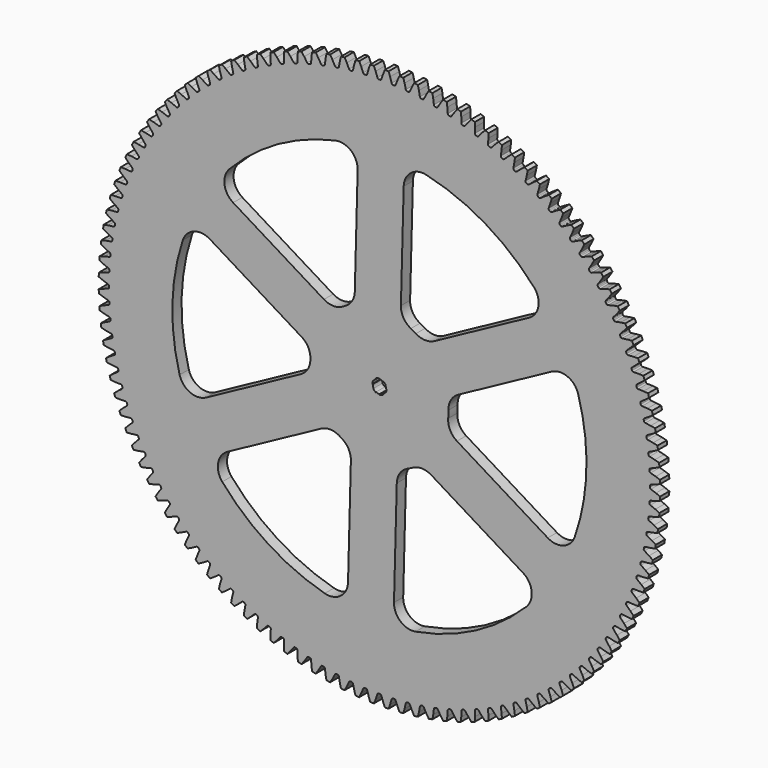
from build123d import *

# Parameters (mm, degrees)
F1_DEPTH = 5


# Not quite as in the source:
# - ends of sketch curves that miss each other by under 0.0002 mm in the source are joined


with BuildPart() as f1:
    # F0 (on Front) → F1 (new body)
    with BuildSketch(Plane.XZ):
        with BuildLine():
            ThreePointArc((12.5188159785, 116.8311997991), (12.2820946911, 116.8563226787), (12.0453229916, 116.8809659184))
            ThreePointArc((12.0453229916, 116.8809659184), (11.6722428914, 117.0473318291), (11.4700517468, 117.4022759484))
            Line((11.4700517468, 117.4022759484), (10.93607, 119.66699))
            Line((10.93607, 119.66699), (10.378861, 121.55772))
            ThreePointArc((10.378861, 121.55772), (9.5720097394, 121.6239147107), (8.7647370086, 121.6847541197))
            Line((8.7647370086, 121.6847541197), (7.918613, 119.904469))
            Line((7.918613, 119.904469), (7.036925, 117.751171))
            ThreePointArc((7.036925, 117.751171), (6.7816984949, 117.4322262933), (6.3871860261, 117.3262704792))
            ThreePointArc((6.3871860261, 117.3262704792), (6.149474622, 117.3389703461), (5.9117380062, 117.3511881224))
            ThreePointArc((5.9117380062, 117.3511881224), (5.5304627311, 117.4978004577), (5.3099725657, 117.8416758875))
            Line((5.3099725657, 117.8416758875), (4.658196, 120.07534))
            Line((4.658196, 120.07534), (4.002798, 121.934317))
            ThreePointArc((4.002798, 121.934317), (3.1935878113, 121.9581936439), (2.3842370057, 121.9767002911))
            Line((2.3842370057, 121.9767002911), (1.632446, 120.154572))
            Line((1.632446, 120.154572), (0.864661, 117.958081))
            ThreePointArc((0.864661, 117.958081), (0.626476604, 117.6262158786), (0.2380500007, 117.4997583469))
            ThreePointArc((0.2380500007, 117.4997583469), (0, 117.5), (-0.2380499997, 117.4997588602))
            ThreePointArc((-0.2380499997, 117.4997588602), (-0.626476604, 117.6262158786), (-0.8646619695, 117.9580810096))
            Line((-0.8646619695, 117.9580810096), (-1.632446, 120.154572))
            Line((-1.632446, 120.154572), (-2.384237, 121.9767))
            ThreePointArc((-2.384237, 121.9767), (-3.1935878113, 121.9581936439), (-4.0027979927, 121.9343167785))
            Line((-4.0027979927, 121.9343167785), (-4.658196, 120.07534))
            Line((-4.658196, 120.07534), (-5.309973, 117.841676))
            ThreePointArc((-5.309973, 117.841676), (-5.5304627311, 117.4978004577), (-5.9117380222, 117.3511874407))
            ThreePointArc((-5.9117380222, 117.3511874407), (-6.149474622, 117.3389703461), (-6.3871859973, 117.32627095))
            ThreePointArc((-6.3871859973, 117.32627095), (-6.7816984949, 117.4322262933), (-7.0369256954, 117.751171114))
            Line((-7.0369256954, 117.751171114), (-7.918613, 119.904469))
            Line((-7.918613, 119.904469), (-8.764737, 121.684754))
            ThreePointArc((-8.764737, 121.684754), (-9.5720097394, 121.6239147107), (-10.3788609835, 121.557719807))
            Line((-10.3788609835, 121.557719807), (-10.93607, 119.66699))
            Line((-10.93607, 119.66699), (-11.470052, 117.402276))
            ThreePointArc((-11.470052, 117.402276), (-11.6722428914, 117.0473318291), (-12.0453230413, 116.8809654005))
            ThreePointArc((-12.0453230413, 116.8809654005), (-12.2820946911, 116.8563226787), (-12.5188159785, 116.8311997991))
            ThreePointArc((-12.5188159785, 116.8311997991), (-12.9183323957, 116.9163625832), (-13.1899018104, 117.2215120825))
            Line((-13.1899018104, 117.2215120825), (-14.183076, 119.325716))
            Line((-14.183076, 119.325716), (-15.121213, 121.059279))
            ThreePointArc((-15.121213, 121.059279), (-15.9241955348, 120.9562730766), (-16.7264769334, 120.8479415191))
            Line((-16.7264769334, 120.8479415191), (-17.183969, 118.930641))
            Line((-17.183969, 118.930641), (-17.598693, 116.641084))
            ThreePointArc((-17.598693, 116.641084), (-17.7820307218, 116.2760450671), (-18.1458920355, 116.0903812274))
            ThreePointArc((-18.1458920355, 116.0903812274), (-18.3810497748, 116.0533799989), (-18.6161320758, 116.0159024726))
            ThreePointArc((-18.6161320758, 116.0159024726), (-19.0195578123, 116.0800394682), (-19.3067252521, 116.3705578742))
            Line((-19.3067252521, 116.3705578742), (-20.408664, 118.419899))
            Line((-20.408664, 118.419899), (-21.436243, 120.101988))
            ThreePointArc((-21.436243, 120.101988), (-22.232733934, 119.9570987554), (-23.0282459144, 119.8069275547))
            Line((-23.0282459144, 119.8069275547), (-23.384768, 117.868311))
            Line((-23.384768, 117.868311), (-23.679098, 115.560187))
            ThreePointArc((-23.679098, 115.560187), (-23.8430793067, 115.1860531874), (-24.1967249351, 114.9816006917))
            ThreePointArc((-24.1967249351, 114.9816006917), (-24.4296235796, 114.9323431057), (-24.6624219479, 114.8826137571))
            ThreePointArc((-24.6624219479, 114.8826137571), (-25.0686523696, 114.925549128), (-25.3706310609, 115.2006409655))
            Line((-25.3706310609, 115.2006409655), (-26.578313, 117.189502))
            Line((-26.578313, 117.189502), (-27.692518, 118.815506))
            ThreePointArc((-27.692518, 118.815506), (-28.4803345272, 118.6291302557), (-29.2668969908, 118.4375309627))
            Line((-29.2668969908, 118.4375309627), (-29.52147, 116.482912))
            Line((-29.52147, 116.482912), (-29.694599, 114.162548))
            ThreePointArc((-29.694599, 114.162548), (-29.8387752501, 113.7803447078), (-30.1812359637, 113.5576638636))
            ThreePointArc((-30.1812359637, 113.5576638636), (-30.4112373541, 113.4962847083), (-30.6411139498, 113.434439814))
            ThreePointArc((-30.6411139498, 113.434439814), (-31.049034801, 113.4560558997), (-31.3649970576, 113.7149659633))
            Line((-31.3649970576, 113.7149659633), (-32.675113, 115.637896))
            Line((-32.675113, 115.637896), (-33.872889, 117.203359))
            ThreePointArc((-33.872889, 117.203359), (-34.6498719533, 116.9760076837), (-35.4253291256, 116.743505414))
            Line((-35.4253291256, 116.743505414), (-35.577257, 114.778242))
            Line((-35.577257, 114.778242), (-35.62871, 112.451997))
            ThreePointArc((-35.62871, 112.451997), (-35.7526848939, 112.0627712751), (-36.0830228615, 111.8224725708))
            ThreePointArc((-36.0830228615, 111.8224725708), (-36.3094969483, 111.7491406292), (-36.5358218851, 111.6753496488))
            ThreePointArc((-36.5358218851, 111.6753496488), (-36.9443140777, 111.675587609), (-37.2733932969, 111.9176057881))
            Line((-37.2733932969, 111.9176057881), (-38.682353, 113.769335))
            Line((-38.682353, 113.769335), (-39.960417, 115.269966))
            ThreePointArc((-39.960417, 115.269966), (-40.7244366229, 115.0022619854), (-41.4866629995, 114.7294939986))
            Line((-41.4866629995, 114.7294939986), (-41.535528, 112.758973))
            Line((-41.535528, 112.758973), (-41.465165, 110.433222))
            ThreePointArc((-41.465165, 110.433222), (-41.5685996289, 110.0380418788), (-41.885908054, 109.7807841415))
            ThreePointArc((-41.885908054, 109.7807841415), (-42.1082339338, 109.6957001663), (-42.3303870998, 109.6101652584))
            ThreePointArc((-42.3303870998, 109.6101652584), (-42.7383321678, 109.589024), (-43.0796267463, 109.8134882019))
            Line((-43.0796267463, 109.8134882019), (-44.583567, 111.588941))
            Line((-44.583567, 111.588941), (-45.938417, 113.020626))
            ThreePointArc((-45.938417, 113.020626), (-46.6873788417, 112.7133029278), (-47.4342849744, 112.4010169392))
            Line((-47.4342849744, 112.4010169392), (-47.379954, 110.430639))
            Line((-47.379954, 110.430639), (-47.187966, 108.111758))
            ThreePointArc((-47.187966, 108.111758), (-47.2705779457, 107.7117061545), (-47.5739877925, 107.4381945315))
            ThreePointArc((-47.5739877925, 107.4381945315), (-47.7915555707, 107.3415912689), (-48.0089271166, 107.2445472605))
            ThreePointArc((-48.0089271166, 107.2445472605), (-48.4152069767, 107.2020847123), (-48.7677816449, 107.4083793144))
            Line((-48.7677816449, 107.4083793144), (-50.362581, 109.102688))
            Line((-50.362581, 109.102688), (-51.790502, 110.461504))
            ThreePointArc((-51.790502, 110.461504), (-52.5223533773, 110.1154048974), (-53.2518919605, 109.7644569186))
            Line((-53.2518919605, 109.7644569186), (-53.094515, 107.799623))
            Line((-53.094515, 107.799623), (-52.781429, 105.493968))
            ThreePointArc((-52.781429, 105.493968), (-52.8429902933, 105.0901404863), (-53.1316701176, 104.8011242319))
            ThreePointArc((-53.1316701176, 104.8011242319), (-53.3438840173, 104.6932664403), (-53.5558789847, 104.5849789701))
            ThreePointArc((-53.5558789847, 104.5849789701), (-53.959379825, 104.5213114069), (-54.3222675686, 104.7088714242))
            Line((-54.3222675686, 104.7088714242), (-56.003554, 106.317393))
            Line((-56.003554, 106.317393), (-57.500634, 107.599615))
            ThreePointArc((-57.500634, 107.599615), (-58.2133685639, 107.2156878467), (-58.9235399183, 106.8270398518))
            Line((-58.9235399183, 106.8270398518), (-58.663547, 104.873135))
            Line((-58.663547, 104.873135), (-58.230222, 102.587025))
            ThreePointArc((-58.230222, 102.587025), (-58.2705637537, 102.180529216), (-58.5437219745, 101.8768009556))
            ThreePointArc((-58.5437219745, 101.8768009556), (-58.7500001006, 101.7579848866), (-58.9560369923, 101.6387509868))
            ThreePointArc((-58.9560369923, 101.6387509868), (-59.3556524519, 101.554053021), (-59.7278592232, 101.7223637563))
            Line((-59.7278592232, 101.7223637563), (-61.491025, 103.240689))
            Line((-61.491025, 103.240689), (-63.05316, 104.442803))
            ThreePointArc((-63.05316, 104.442803), (-63.7448248599, 104.0221000729), (-64.4336830055, 103.5968170088))
            Line((-64.4336830055, 103.5968170088), (-64.071786, 101.659197))
            Line((-64.071786, 101.659197), (-63.519409, 99.398899))
            ThreePointArc((-63.519409, 99.398899), (-63.5384209901, 98.9908485982), (-63.7953090424, 98.6732400656))
            ThreePointArc((-63.7953090424, 98.6732400656), (-63.9950864156, 98.5437918626), (-64.1946010227, 98.4139380349))
            ThreePointArc((-64.1946010227, 98.4139380349), (-64.5892361181, 98.3084414707), (-64.9697412666, 98.4570416764))
            Line((-64.9697412666, 98.4570416764), (-66.809954, 99.88101))
            Line((-66.809954, 99.88101), (-68.432862, 100.99972))
            ThreePointArc((-68.432862, 100.99972), (-69.1015608372, 100.5433950583), (-69.7672170052, 100.0826430074))
            Line((-69.7672170052, 100.0826430074), (-69.304409, 98.166618))
            Line((-69.304409, 98.166618), (-68.634495, 95.938327))
            ThreePointArc((-68.634495, 95.938327), (-68.6321244527, 95.5298408511), (-68.8720381709, 95.1992232362))
            ThreePointArc((-68.8720381709, 95.1992232362), (-69.0647673265, 95.0594967068), (-69.2572121912, 94.9193792621))
            ThreePointArc((-69.2572121912, 94.9193792621), (-69.6457852997, 94.7933743382), (-70.03354633, 94.9218565538))
            Line((-70.03354633, 94.9218565538), (-71.945762, 96.247563))
            Line((-71.945762, 96.247563), (-73.624994, 97.279804))
            ThreePointArc((-73.624994, 97.279804), (-74.2688945566, 96.7891073486), (-74.9095248305, 96.2941487821))
            Line((-74.9095248305, 96.2941487821), (-74.347074, 94.404972))
            Line((-74.347074, 94.404972), (-73.561458, 92.214795))
            ThreePointArc((-73.561458, 92.214795), (-73.5377128489, 91.8069932074), (-73.7599940376, 91.4642730467))
            ThreePointArc((-73.7599940376, 91.4642730467), (-73.9451458655, 91.3146505383), (-74.1299940885, 91.1646531088))
            ThreePointArc((-74.1299940885, 91.1646531088), (-74.5114399991, 91.0184844006), (-74.9053938653, 91.1264972037))
            Line((-74.9053938653, 91.1264972037), (-76.884371, 92.350309))
            Line((-76.884371, 92.350309), (-78.615325, 93.293251))
            ThreePointArc((-78.615325, 93.293251), (-79.2326618352, 92.7695278554), (-79.8465098183, 92.2417197901))
            Line((-79.8465098183, 92.2417197901), (-79.185958, 90.384568))
            Line((-79.185958, 90.384568), (-78.286794, 88.238509))
            ThreePointArc((-78.286794, 88.238509), (-78.2417385737, 87.8325087165), (-78.445778564, 87.4786245138))
            ThreePointArc((-78.445778564, 87.4786245138), (-78.6228462028, 87.3195170336), (-78.7995909084, 87.1600508987))
            ThreePointArc((-78.7995909084, 87.1600508987), (-79.1728641926, 86.9941195101), (-79.57193092, 87.0813661359))
            Line((-79.57193092, 87.0813661359), (-81.612245, 88.199929))
            Line((-81.612245, 88.199929), (-83.390177, 89.050988))
            ThreePointArc((-83.390177, 89.050988), (-83.979258287, 88.4956732138), (-84.5646419271, 87.9364619242))
            Line((-84.5646419271, 87.9364619242), (-83.8078, 86.116426))
            Line((-83.8078, 86.116426), (-82.797551, 84.020367))
            ThreePointArc((-82.797551, 84.020367), (-82.7313095419, 83.6172808287), (-82.9165489842, 83.2532029842))
            ThreePointArc((-82.9165489842, 83.2532029842), (-83.0850467894, 83.0850467894), (-83.2532032779, 82.9165492768))
            ThreePointArc((-83.2532032779, 82.9165492768), (-83.6172808287, 82.7313095419), (-84.0203668833, 82.7975512243))
            Line((-84.0203668833, 82.7975512243), (-86.116426, 83.8078))
            Line((-86.116426, 83.8078), (-87.936462, 84.564642))
            ThreePointArc((-87.936462, 84.564642), (-88.4956732138, 83.979258287), (-89.0509877491, 83.3901767651))
            Line((-89.0509877491, 83.3901767651), (-88.199929, 81.612245))
            Line((-88.199929, 81.612245), (-87.081366, 79.571931))
            ThreePointArc((-87.081366, 79.571931), (-86.9941195101, 79.1728641926), (-87.1600507346, 78.7995907601))
            ThreePointArc((-87.1600507346, 78.7995907601), (-87.3195170336, 78.6228462028), (-87.478624763, 78.4457787875))
            ThreePointArc((-87.478624763, 78.4457787875), (-87.8325087165, 78.2417385737), (-88.2385092035, 78.2867935531))
            Line((-88.2385092035, 78.2867935531), (-90.384568, 79.185958))
            Line((-90.384568, 79.185958), (-92.24172, 79.84651))
            ThreePointArc((-92.24172, 79.84651), (-92.7695278554, 79.2326618352), (-93.293250978, 78.6153249815))
            Line((-93.293250978, 78.6153249815), (-92.350309, 76.884371))
            Line((-92.350309, 76.884371), (-91.126497, 74.905394))
            ThreePointArc((-91.126497, 74.905394), (-91.0184844006, 74.5114399991), (-91.1646526812, 74.1299937408))
            ThreePointArc((-91.1646526812, 74.1299937408), (-91.3146505383, 73.9451458655), (-91.4642731646, 73.7599941328))
            ThreePointArc((-91.4642731646, 73.7599941328), (-91.8069932074, 73.5377128489), (-92.2147949261, 73.5614571878))
            Line((-92.2147949261, 73.5614571878), (-94.404972, 74.347074))
            Line((-94.404972, 74.347074), (-96.294149, 74.909525))
            ThreePointArc((-96.294149, 74.909525), (-96.7891073486, 74.2688945566), (-97.2798039746, 73.6249939808))
            Line((-97.2798039746, 73.6249939808), (-96.247563, 71.945762))
            Line((-96.247563, 71.945762), (-94.921857, 70.033546))
            ThreePointArc((-94.921857, 70.033546), (-94.7933743382, 69.6457852997), (-94.9193792786, 69.2572122033))
            ThreePointArc((-94.9193792786, 69.2572122033), (-95.0594967068, 69.0647673265), (-95.1992239786, 68.8720389845))
            ThreePointArc((-95.1992239786, 68.8720389845), (-95.5298408511, 68.6321244527), (-95.9383270634, 68.6344938104))
            Line((-95.9383270634, 68.6344938104), (-98.166618, 69.304409))
            Line((-98.166618, 69.304409), (-100.082643, 69.767217))
            ThreePointArc((-100.082643, 69.767217), (-100.5433950583, 69.1015608372), (-100.9997198589, 68.4328619044))
            Line((-100.9997198589, 68.4328619044), (-99.88101, 66.809954))
            Line((-99.88101, 66.809954), (-98.457042, 64.969741))
            ThreePointArc((-98.457042, 64.969741), (-98.3084414707, 64.5892361181), (-98.4139369801, 64.194600987))
            ThreePointArc((-98.4139369801, 64.194600987), (-98.5437918626, 63.9950864156), (-98.6732412149, 63.795309139))
            ThreePointArc((-98.6732412149, 63.795309139), (-98.9908485982, 63.5384209901), (-99.3988990683, 63.5194087532))
            Line((-99.3988990683, 63.5194087532), (-101.659197, 64.071786))
            Line((-101.659197, 64.071786), (-103.596817, 64.433683))
            ThreePointArc((-103.596817, 64.433683), (-104.0221000729, 63.7448248599), (-104.4428027036, 63.0531598211))
            Line((-104.4428027036, 63.0531598211), (-103.240689, 61.491025))
            Line((-103.240689, 61.491025), (-101.722364, 59.727859))
            ThreePointArc((-101.722364, 59.727859), (-101.554053021, 59.3556524519), (-101.6387505676, 58.9560367492))
            ThreePointArc((-101.6387505676, 58.9560367492), (-101.7579848866, 58.7500001006), (-101.8768011195, 58.5437220687))
            ThreePointArc((-101.8768011195, 58.5437220687), (-102.180529216, 58.2705637537), (-102.5870249232, 58.2302213469))
            Line((-102.5870249232, 58.2302213469), (-104.873135, 58.663547))
            Line((-104.873135, 58.663547), (-106.82704, 58.92354))
            ThreePointArc((-106.82704, 58.92354), (-107.2156878467, 58.2133685639), (-107.5996147884, 57.5006338869))
            Line((-107.5996147884, 57.5006338869), (-106.317393, 56.003554))
            Line((-106.317393, 56.003554), (-104.708872, 54.322267))
            ThreePointArc((-104.708872, 54.322267), (-104.5213114069, 53.959379825), (-104.5849782669, 53.5558791367))
            ThreePointArc((-104.5849782669, 53.5558791367), (-104.6932664403, 53.3438840173), (-104.8011241949, 53.1316700988))
            ThreePointArc((-104.8011241949, 53.1316700988), (-105.0901404863, 52.8429902933), (-105.4939679887, 52.7814290678))
            Line((-105.4939679887, 52.7814290678), (-107.799623, 53.094515))
            Line((-107.799623, 53.094515), (-109.764457, 53.251892))
            ThreePointArc((-109.764457, 53.251892), (-110.1154048974, 52.5223533773), (-110.461504136, 51.7905020638))
            Line((-110.461504136, 51.7905020638), (-109.102688, 50.362581))
            Line((-109.102688, 50.362581), (-107.40838, 48.767781))
            ThreePointArc((-107.40838, 48.767781), (-107.2020847123, 48.4152069767), (-107.2445473797, 48.00892717))
            ThreePointArc((-107.2445473797, 48.00892717), (-107.3415912689, 47.7915555707), (-107.4381946923, 47.5739878637))
            ThreePointArc((-107.4381946923, 47.5739878637), (-107.7117061545, 47.2705779457), (-108.1117579692, 47.1879662713))
            Line((-108.1117579692, 47.1879662713), (-110.430639, 47.379954))
            Line((-110.430639, 47.379954), (-112.401017, 47.434285))
            ThreePointArc((-112.401017, 47.434285), (-112.7133029278, 46.6873788417), (-113.0206257802, 45.9384169107))
            Line((-113.0206257802, 45.9384169107), (-111.588941, 44.583567))
            Line((-111.588941, 44.583567), (-109.813489, 43.079626))
            ThreePointArc((-109.813489, 43.079626), (-109.589024, 42.7383321678), (-109.6101651266, 42.3303870489))
            ThreePointArc((-109.6101651266, 42.3303870489), (-109.6957001663, 42.1082339338), (-109.7807848243, 41.885907933))
            ThreePointArc((-109.7807848243, 41.885907933), (-110.0380418788, 41.5685996289), (-110.4332219815, 41.4651643038))
            Line((-110.4332219815, 41.4651643038), (-112.758973, 41.535528))
            Line((-112.758973, 41.535528), (-114.729494, 41.486663))
            ThreePointArc((-114.729494, 41.486663), (-115.0022619854, 40.7244366229), (-115.2699660447, 39.9604170155))
            Line((-115.2699660447, 39.9604170155), (-113.769335, 38.682353))
            Line((-113.769335, 38.682353), (-111.917606, 37.273393))
            ThreePointArc((-111.917606, 37.273393), (-111.675587609, 36.9443140777), (-111.6753496356, 36.5358218808))
            ThreePointArc((-111.6753496356, 36.5358218808), (-111.7491406292, 36.3094969483), (-111.8224729326, 36.0830229782))
            ThreePointArc((-111.8224729326, 36.0830229782), (-112.0627712751, 35.7526848939), (-112.4519969984, 35.6287091852))
            Line((-112.4519969984, 35.6287091852), (-114.778242, 35.577257))
            Line((-114.778242, 35.577257), (-116.743505, 35.425329))
            ThreePointArc((-116.743505, 35.425329), (-116.9760076837, 34.6498719533), (-117.2033591178, 33.872889034))
            Line((-117.2033591178, 33.872889034), (-115.637896, 32.675113))
            Line((-115.637896, 32.675113), (-113.714966, 31.364997))
            ThreePointArc((-113.714966, 31.364997), (-113.4560558997, 31.049034801), (-113.4344393857, 30.6411141042))
            ThreePointArc((-113.4344393857, 30.6411141042), (-113.4962847083, 30.4112373541), (-113.5576637548, 30.1812359348))
            ThreePointArc((-113.5576637548, 30.1812359348), (-113.7803447078, 29.8387752501), (-114.1625480084, 29.6945991918))
            Line((-114.1625480084, 29.6945991918), (-116.482912, 29.52147))
            Line((-116.482912, 29.52147), (-118.437531, 29.266897))
            ThreePointArc((-118.437531, 29.266897), (-118.6291302557, 28.4803345272), (-118.8155059233, 27.6925179821))
            Line((-118.8155059233, 27.6925179821), (-117.189502, 26.578313))
            Line((-117.189502, 26.578313), (-115.200641, 25.37063))
            ThreePointArc((-115.200641, 25.37063), (-114.925549128, 25.0686523696), (-114.8826129045, 24.6624219795))
            ThreePointArc((-114.8826129045, 24.6624219795), (-114.9323431057, 24.4296235796), (-114.9816007116, 24.1967249393))
            ThreePointArc((-114.9816007116, 24.1967249393), (-115.1860531874, 23.8430793067), (-115.5601869717, 23.6790977072))
            Line((-115.5601869717, 23.6790977072), (-117.868311, 23.384768))
            Line((-117.868311, 23.384768), (-119.806927, 23.028246))
            ThreePointArc((-119.806927, 23.028246), (-119.9570987554, 22.232733934), (-120.1019878567, 21.4362429744))
            Line((-120.1019878567, 21.4362429744), (-118.419899, 20.408664))
            Line((-118.419899, 20.408664), (-116.370558, 19.306725))
            ThreePointArc((-116.370558, 19.306725), (-116.0800394682, 19.0195578123), (-116.0159016824, 18.616131949))
            ThreePointArc((-116.0159016824, 18.616131949), (-116.0533799989, 18.3810497748), (-116.0903811799, 18.1458920281))
            ThreePointArc((-116.0903811799, 18.1458920281), (-116.2760450671, 17.7820307218), (-116.641084015, 17.5986931001))
            Line((-116.641084015, 17.5986931001), (-118.930641, 17.183969))
            Line((-118.930641, 17.183969), (-120.847942, 16.726477))
            ThreePointArc((-120.847942, 16.726477), (-120.9562730766, 15.9241955348), (-121.059278534, 15.1212129418))
            Line((-121.059278534, 15.1212129418), (-119.325716, 14.183076))
            Line((-119.325716, 14.183076), (-117.221512, 13.189902))
            ThreePointArc((-117.221512, 13.189902), (-116.9163625832, 12.9183323957), (-116.8311990873, 12.5188160094))
            ThreePointArc((-116.8311990873, 12.5188160094), (-116.8563226787, 12.2820946911), (-116.8809659184, 12.0453229916))
            ThreePointArc((-116.8809659184, 12.0453229916), (-117.0473318291, 11.6722428914), (-117.4022759484, 11.4700517468))
            Line((-117.4022759484, 11.4700517468), (-119.66699, 10.93607))
            Line((-119.66699, 10.93607), (-121.55772, 10.378861))
            ThreePointArc((-121.55772, 10.378861), (-121.6239147107, 9.5720097394), (-121.6847541197, 8.7647370086))
            Line((-121.6847541197, 8.7647370086), (-119.904469, 7.918613))
            Line((-119.904469, 7.918613), (-117.751171, 7.036925))
            ThreePointArc((-117.751171, 7.036925), (-117.4322262933, 6.7816984949), (-117.3262704792, 6.3871860261))
            ThreePointArc((-117.3262704792, 6.3871860261), (-117.3389703461, 6.149474622), (-117.3511881224, 5.9117380062))
            ThreePointArc((-117.3511881224, 5.9117380062), (-117.4978004577, 5.5304627311), (-117.8416758875, 5.3099725657))
            Line((-117.8416758875, 5.3099725657), (-120.07534, 4.658196))
            Line((-120.07534, 4.658196), (-121.934317, 4.002798))
            ThreePointArc((-121.934317, 4.002798), (-121.9581936439, 3.1935878113), (-121.9767002911, 2.3842370057))
            Line((-121.9767002911, 2.3842370057), (-120.154572, 1.632446))
            Line((-120.154572, 1.632446), (-117.958081, 0.864661))
            ThreePointArc((-117.958081, 0.864661), (-117.6262158786, 0.626476604), (-117.4997583469, 0.2380500007))
            ThreePointArc((-117.4997583469, 0.2380500007), (-117.5, 0), (-117.4997588602, -0.2380499997))
            ThreePointArc((-117.4997588602, -0.2380499997), (-117.6262158786, -0.626476604), (-117.9580810096, -0.8646619695))
            Line((-117.9580810096, -0.8646619695), (-120.154572, -1.632446))
            Line((-120.154572, -1.632446), (-121.9767, -2.384237))
            ThreePointArc((-121.9767, -2.384237), (-121.9581936439, -3.1935878113), (-121.9343167785, -4.0027979927))
            Line((-121.9343167785, -4.0027979927), (-120.07534, -4.658196))
            Line((-120.07534, -4.658196), (-117.841676, -5.309973))
            ThreePointArc((-117.841676, -5.309973), (-117.4978004577, -5.5304627311), (-117.3511874407, -5.9117380222))
            ThreePointArc((-117.3511874407, -5.9117380222), (-117.3389703461, -6.149474622), (-117.32627095, -6.3871859973))
            ThreePointArc((-117.32627095, -6.3871859973), (-117.4322262933, -6.7816984949), (-117.751171114, -7.0369256954))
            Line((-117.751171114, -7.0369256954), (-119.904469, -7.918613))
            Line((-119.904469, -7.918613), (-121.684754, -8.764737))
            ThreePointArc((-121.684754, -8.764737), (-121.6239147107, -9.5720097394), (-121.557719807, -10.3788609835))
            Line((-121.557719807, -10.3788609835), (-119.66699, -10.93607))
            Line((-119.66699, -10.93607), (-117.402276, -11.470052))
            ThreePointArc((-117.402276, -11.470052), (-117.0473318291, -11.6722428914), (-116.8809654005, -12.0453230413))
            ThreePointArc((-116.8809654005, -12.0453230413), (-116.8563226787, -12.2820946911), (-116.8311997991, -12.5188159785))
            ThreePointArc((-116.8311997991, -12.5188159785), (-116.9163625832, -12.9183323957), (-117.2215120825, -13.1899018104))
            Line((-117.2215120825, -13.1899018104), (-119.325716, -14.183076))
            Line((-119.325716, -14.183076), (-121.059279, -15.121213))
            ThreePointArc((-121.059279, -15.121213), (-120.9562730766, -15.9241955348), (-120.8479415191, -16.7264769334))
            Line((-120.8479415191, -16.7264769334), (-118.930641, -17.183969))
            Line((-118.930641, -17.183969), (-116.641084, -17.598693))
            ThreePointArc((-116.641084, -17.598693), (-116.2760450671, -17.7820307218), (-116.0903812274, -18.1458920355))
            ThreePointArc((-116.0903812274, -18.1458920355), (-116.0533799989, -18.3810497748), (-116.0159024726, -18.6161320758))
            ThreePointArc((-116.0159024726, -18.6161320758), (-116.0800394682, -19.0195578123), (-116.3705578742, -19.3067252521))
            Line((-116.3705578742, -19.3067252521), (-118.419899, -20.408664))
            Line((-118.419899, -20.408664), (-120.101988, -21.436243))
            ThreePointArc((-120.101988, -21.436243), (-119.9570987554, -22.232733934), (-119.8069275547, -23.0282459144))
            Line((-119.8069275547, -23.0282459144), (-117.868311, -23.384768))
            Line((-117.868311, -23.384768), (-115.560187, -23.679098))
            ThreePointArc((-115.560187, -23.679098), (-115.1860531874, -23.8430793067), (-114.9816006917, -24.1967249351))
            ThreePointArc((-114.9816006917, -24.1967249351), (-114.9323431057, -24.4296235796), (-114.8826137571, -24.6624219479))
            ThreePointArc((-114.8826137571, -24.6624219479), (-114.925549128, -25.0686523696), (-115.2006409655, -25.3706310609))
            Line((-115.2006409655, -25.3706310609), (-117.189502, -26.578313))
            Line((-117.189502, -26.578313), (-118.815506, -27.692518))
            ThreePointArc((-118.815506, -27.692518), (-118.6291302557, -28.4803345272), (-118.4375309627, -29.2668969908))
            Line((-118.4375309627, -29.2668969908), (-116.482912, -29.52147))
            Line((-116.482912, -29.52147), (-114.162548, -29.694599))
            ThreePointArc((-114.162548, -29.694599), (-113.7803447078, -29.8387752501), (-113.5576638636, -30.1812359637))
            ThreePointArc((-113.5576638636, -30.1812359637), (-113.4962847083, -30.4112373541), (-113.434439814, -30.6411139498))
            ThreePointArc((-113.434439814, -30.6411139498), (-113.4560558997, -31.049034801), (-113.7149659633, -31.3649970576))
            Line((-113.7149659633, -31.3649970576), (-115.637896, -32.675113))
            Line((-115.637896, -32.675113), (-117.203359, -33.872889))
            ThreePointArc((-117.203359, -33.872889), (-116.9760076837, -34.6498719533), (-116.743505414, -35.4253291256))
            Line((-116.743505414, -35.4253291256), (-114.778242, -35.577257))
            Line((-114.778242, -35.577257), (-112.451997, -35.62871))
            ThreePointArc((-112.451997, -35.62871), (-112.0627712751, -35.7526848939), (-111.8224725708, -36.0830228615))
            ThreePointArc((-111.8224725708, -36.0830228615), (-111.7491406292, -36.3094969483), (-111.6753496488, -36.5358218851))
            ThreePointArc((-111.6753496488, -36.5358218851), (-111.675587609, -36.9443140777), (-111.9176057881, -37.2733932969))
            Line((-111.9176057881, -37.2733932969), (-113.769335, -38.682353))
            Line((-113.769335, -38.682353), (-115.269966, -39.960417))
            ThreePointArc((-115.269966, -39.960417), (-115.0022619854, -40.7244366229), (-114.7294939986, -41.4866629995))
            Line((-114.7294939986, -41.4866629995), (-112.758973, -41.535528))
            Line((-112.758973, -41.535528), (-110.433222, -41.465165))
            ThreePointArc((-110.433222, -41.465165), (-110.0380418788, -41.5685996289), (-109.7807841415, -41.885908054))
            ThreePointArc((-109.7807841415, -41.885908054), (-109.6957001663, -42.1082339338), (-109.6101652584, -42.3303870998))
            ThreePointArc((-109.6101652584, -42.3303870998), (-109.589024, -42.7383321678), (-109.8134882019, -43.0796267463))
            Line((-109.8134882019, -43.0796267463), (-111.588941, -44.583567))
            Line((-111.588941, -44.583567), (-113.020626, -45.938417))
            ThreePointArc((-113.020626, -45.938417), (-112.7133029278, -46.6873788417), (-112.4010169392, -47.4342849744))
            Line((-112.4010169392, -47.4342849744), (-110.430639, -47.379954))
            Line((-110.430639, -47.379954), (-108.111758, -47.187966))
            ThreePointArc((-108.111758, -47.187966), (-107.7117061545, -47.2705779457), (-107.4381945315, -47.5739877925))
            ThreePointArc((-107.4381945315, -47.5739877925), (-107.3415912689, -47.7915555707), (-107.2445472605, -48.0089271166))
            ThreePointArc((-107.2445472605, -48.0089271166), (-107.2020847123, -48.4152069767), (-107.4083793144, -48.7677816449))
            Line((-107.4083793144, -48.7677816449), (-109.102688, -50.362581))
            Line((-109.102688, -50.362581), (-110.461504, -51.790502))
            ThreePointArc((-110.461504, -51.790502), (-110.1154048974, -52.5223533773), (-109.7644569186, -53.2518919605))
            Line((-109.7644569186, -53.2518919605), (-107.799623, -53.094515))
            Line((-107.799623, -53.094515), (-105.493968, -52.781429))
            ThreePointArc((-105.493968, -52.781429), (-105.0901404863, -52.8429902933), (-104.8011242319, -53.1316701176))
            ThreePointArc((-104.8011242319, -53.1316701176), (-104.6932664403, -53.3438840173), (-104.5849789701, -53.5558789847))
            ThreePointArc((-104.5849789701, -53.5558789847), (-104.5213114069, -53.959379825), (-104.7088714242, -54.3222675686))
            Line((-104.7088714242, -54.3222675686), (-106.317393, -56.003554))
            Line((-106.317393, -56.003554), (-107.599615, -57.500634))
            ThreePointArc((-107.599615, -57.500634), (-107.2156878467, -58.2133685639), (-106.8270398518, -58.9235399183))
            Line((-106.8270398518, -58.9235399183), (-104.873135, -58.663547))
            Line((-104.873135, -58.663547), (-102.587025, -58.230222))
            ThreePointArc((-102.587025, -58.230222), (-102.180529216, -58.2705637537), (-101.8768009556, -58.5437219745))
            ThreePointArc((-101.8768009556, -58.5437219745), (-101.7579848866, -58.7500001006), (-101.6387509868, -58.9560369923))
            ThreePointArc((-101.6387509868, -58.9560369923), (-101.554053021, -59.3556524519), (-101.7223637563, -59.7278592232))
            Line((-101.7223637563, -59.7278592232), (-103.240689, -61.491025))
            Line((-103.240689, -61.491025), (-104.442803, -63.05316))
            ThreePointArc((-104.442803, -63.05316), (-104.0221000729, -63.7448248599), (-103.5968170088, -64.4336830055))
            Line((-103.5968170088, -64.4336830055), (-101.659197, -64.071786))
            Line((-101.659197, -64.071786), (-99.398899, -63.519409))
            ThreePointArc((-99.398899, -63.519409), (-98.9908485982, -63.5384209901), (-98.6732400656, -63.7953090424))
            ThreePointArc((-98.6732400656, -63.7953090424), (-98.5437918626, -63.9950864156), (-98.4139380349, -64.1946010227))
            ThreePointArc((-98.4139380349, -64.1946010227), (-98.3084414707, -64.5892361181), (-98.4570416764, -64.9697412666))
            Line((-98.4570416764, -64.9697412666), (-99.88101, -66.809954))
            Line((-99.88101, -66.809954), (-100.99972, -68.432862))
            ThreePointArc((-100.99972, -68.432862), (-100.5433950583, -69.1015608372), (-100.0826430074, -69.7672170052))
            Line((-100.0826430074, -69.7672170052), (-98.166618, -69.304409))
            Line((-98.166618, -69.304409), (-95.938327, -68.634495))
            ThreePointArc((-95.938327, -68.634495), (-95.5298408511, -68.6321244527), (-95.1992232362, -68.8720381709))
            ThreePointArc((-95.1992232362, -68.8720381709), (-95.0594967068, -69.0647673265), (-94.9193792621, -69.2572121912))
            ThreePointArc((-94.9193792621, -69.2572121912), (-94.7933743382, -69.6457852997), (-94.9218565538, -70.03354633))
            Line((-94.9218565538, -70.03354633), (-96.247563, -71.945762))
            Line((-96.247563, -71.945762), (-97.279804, -73.624994))
            ThreePointArc((-97.279804, -73.624994), (-96.7891073486, -74.2688945566), (-96.2941487821, -74.9095248305))
            Line((-96.2941487821, -74.9095248305), (-94.404972, -74.347074))
            Line((-94.404972, -74.347074), (-92.214795, -73.561458))
            ThreePointArc((-92.214795, -73.561458), (-91.8069932074, -73.5377128489), (-91.4642730467, -73.7599940376))
            ThreePointArc((-91.4642730467, -73.7599940376), (-91.3146505383, -73.9451458655), (-91.1646531088, -74.1299940885))
            ThreePointArc((-91.1646531088, -74.1299940885), (-91.0184844006, -74.5114399991), (-91.1264972037, -74.9053938653))
            Line((-91.1264972037, -74.9053938653), (-92.350309, -76.884371))
            Line((-92.350309, -76.884371), (-93.293251, -78.615325))
            ThreePointArc((-93.293251, -78.615325), (-92.7695278554, -79.2326618352), (-92.2417197901, -79.8465098183))
            Line((-92.2417197901, -79.8465098183), (-90.384568, -79.185958))
            Line((-90.384568, -79.185958), (-88.238509, -78.286794))
            ThreePointArc((-88.238509, -78.286794), (-87.8325087165, -78.2417385737), (-87.4786245138, -78.445778564))
            ThreePointArc((-87.4786245138, -78.445778564), (-87.3195170336, -78.6228462028), (-87.1600508987, -78.7995909084))
            ThreePointArc((-87.1600508987, -78.7995909084), (-86.9941195101, -79.1728641926), (-87.0813661359, -79.57193092))
            Line((-87.0813661359, -79.57193092), (-88.199929, -81.612245))
            Line((-88.199929, -81.612245), (-89.050988, -83.390177))
            ThreePointArc((-89.050988, -83.390177), (-88.4956732138, -83.979258287), (-87.9364619242, -84.5646419271))
            Line((-87.9364619242, -84.5646419271), (-86.116426, -83.8078))
            Line((-86.116426, -83.8078), (-84.020367, -82.797551))
            ThreePointArc((-84.020367, -82.797551), (-83.6172808287, -82.7313095419), (-83.2532029842, -82.9165489842))
            ThreePointArc((-83.2532029842, -82.9165489842), (-83.0850467894, -83.0850467894), (-82.9165492768, -83.2532032779))
            ThreePointArc((-82.9165492768, -83.2532032779), (-82.7313095419, -83.6172808287), (-82.7975512243, -84.0203668833))
            Line((-82.7975512243, -84.0203668833), (-83.8078, -86.116426))
            Line((-83.8078, -86.116426), (-84.564642, -87.936462))
            ThreePointArc((-84.564642, -87.936462), (-83.979258287, -88.4956732138), (-83.3901767651, -89.0509877491))
            Line((-83.3901767651, -89.0509877491), (-81.612245, -88.199929))
            Line((-81.612245, -88.199929), (-79.571931, -87.081366))
            ThreePointArc((-79.571931, -87.081366), (-79.1728641926, -86.9941195101), (-78.7995907601, -87.1600507346))
            ThreePointArc((-78.7995907601, -87.1600507346), (-78.6228462028, -87.3195170336), (-78.4457787875, -87.478624763))
            ThreePointArc((-78.4457787875, -87.478624763), (-78.2417385737, -87.8325087165), (-78.2867935531, -88.2385092035))
            Line((-78.2867935531, -88.2385092035), (-79.185958, -90.384568))
            Line((-79.185958, -90.384568), (-79.84651, -92.24172))
            ThreePointArc((-79.84651, -92.24172), (-79.2326618352, -92.7695278554), (-78.6153249815, -93.293250978))
            Line((-78.6153249815, -93.293250978), (-76.884371, -92.350309))
            Line((-76.884371, -92.350309), (-74.905394, -91.126497))
            ThreePointArc((-74.905394, -91.126497), (-74.5114399991, -91.0184844006), (-74.1299937408, -91.1646526812))
            ThreePointArc((-74.1299937408, -91.1646526812), (-73.9451458655, -91.3146505383), (-73.7599941328, -91.4642731646))
            ThreePointArc((-73.7599941328, -91.4642731646), (-73.5377128489, -91.8069932074), (-73.5614571878, -92.2147949261))
            Line((-73.5614571878, -92.2147949261), (-74.347074, -94.404972))
            Line((-74.347074, -94.404972), (-74.909525, -96.294149))
            ThreePointArc((-74.909525, -96.294149), (-74.2688945566, -96.7891073486), (-73.6249939808, -97.2798039746))
            Line((-73.6249939808, -97.2798039746), (-71.945762, -96.247563))
            Line((-71.945762, -96.247563), (-70.033546, -94.921857))
            ThreePointArc((-70.033546, -94.921857), (-69.6457852997, -94.7933743382), (-69.2572122033, -94.9193792786))
            ThreePointArc((-69.2572122033, -94.9193792786), (-69.0647673265, -95.0594967068), (-68.8720389845, -95.1992239786))
            ThreePointArc((-68.8720389845, -95.1992239786), (-68.6321244527, -95.5298408511), (-68.6344938104, -95.9383270634))
            Line((-68.6344938104, -95.9383270634), (-69.304409, -98.166618))
            Line((-69.304409, -98.166618), (-69.767217, -100.082643))
            ThreePointArc((-69.767217, -100.082643), (-69.1015608372, -100.5433950583), (-68.4328619044, -100.9997198589))
            Line((-68.4328619044, -100.9997198589), (-66.809954, -99.88101))
            Line((-66.809954, -99.88101), (-64.969741, -98.457042))
            ThreePointArc((-64.969741, -98.457042), (-64.5892361181, -98.3084414707), (-64.194600987, -98.4139369801))
            ThreePointArc((-64.194600987, -98.4139369801), (-63.9950864156, -98.5437918626), (-63.795309139, -98.6732412149))
            ThreePointArc((-63.795309139, -98.6732412149), (-63.5384209901, -98.9908485982), (-63.5194087532, -99.3988990683))
            Line((-63.5194087532, -99.3988990683), (-64.071786, -101.659197))
            Line((-64.071786, -101.659197), (-64.433683, -103.596817))
            ThreePointArc((-64.433683, -103.596817), (-63.7448248599, -104.0221000729), (-63.0531598211, -104.4428027036))
            Line((-63.0531598211, -104.4428027036), (-61.491025, -103.240689))
            Line((-61.491025, -103.240689), (-59.727859, -101.722364))
            ThreePointArc((-59.727859, -101.722364), (-59.3556524519, -101.554053021), (-58.9560367492, -101.6387505676))
            ThreePointArc((-58.9560367492, -101.6387505676), (-58.7500001006, -101.7579848866), (-58.5437220687, -101.8768011195))
            ThreePointArc((-58.5437220687, -101.8768011195), (-58.2705637537, -102.180529216), (-58.2302213469, -102.5870249232))
            Line((-58.2302213469, -102.5870249232), (-58.663547, -104.873135))
            Line((-58.663547, -104.873135), (-58.92354, -106.82704))
            ThreePointArc((-58.92354, -106.82704), (-58.2133685639, -107.2156878467), (-57.5006338869, -107.5996147884))
            Line((-57.5006338869, -107.5996147884), (-56.003554, -106.317393))
            Line((-56.003554, -106.317393), (-54.322267, -104.708872))
            ThreePointArc((-54.322267, -104.708872), (-53.959379825, -104.5213114069), (-53.5558791367, -104.5849782669))
            ThreePointArc((-53.5558791367, -104.5849782669), (-53.3438840173, -104.6932664403), (-53.1316700988, -104.8011241949))
            ThreePointArc((-53.1316700988, -104.8011241949), (-52.8429902933, -105.0901404863), (-52.7814290678, -105.4939679887))
            Line((-52.7814290678, -105.4939679887), (-53.094515, -107.799623))
            Line((-53.094515, -107.799623), (-53.251892, -109.764457))
            ThreePointArc((-53.251892, -109.764457), (-52.5223533773, -110.1154048974), (-51.7905020638, -110.461504136))
            Line((-51.7905020638, -110.461504136), (-50.362581, -109.102688))
            Line((-50.362581, -109.102688), (-48.767781, -107.40838))
            ThreePointArc((-48.767781, -107.40838), (-48.4152069767, -107.2020847123), (-48.00892717, -107.2445473797))
            ThreePointArc((-48.00892717, -107.2445473797), (-47.7915555707, -107.3415912689), (-47.5739878637, -107.4381946923))
            ThreePointArc((-47.5739878637, -107.4381946923), (-47.2705779457, -107.7117061545), (-47.1879662713, -108.1117579692))
            Line((-47.1879662713, -108.1117579692), (-47.379954, -110.430639))
            Line((-47.379954, -110.430639), (-47.434285, -112.401017))
            ThreePointArc((-47.434285, -112.401017), (-46.6873788417, -112.7133029278), (-45.9384169107, -113.0206257802))
            Line((-45.9384169107, -113.0206257802), (-44.583567, -111.588941))
            Line((-44.583567, -111.588941), (-43.079626, -109.813489))
            ThreePointArc((-43.079626, -109.813489), (-42.7383321678, -109.589024), (-42.3303870489, -109.6101651266))
            ThreePointArc((-42.3303870489, -109.6101651266), (-42.1082339338, -109.6957001663), (-41.885907933, -109.7807848243))
            ThreePointArc((-41.885907933, -109.7807848243), (-41.5685996289, -110.0380418788), (-41.4651643038, -110.4332219815))
            Line((-41.4651643038, -110.4332219815), (-41.535528, -112.758973))
            Line((-41.535528, -112.758973), (-41.486663, -114.729494))
            ThreePointArc((-41.486663, -114.729494), (-40.7244366229, -115.0022619854), (-39.9604170155, -115.2699660447))
            Line((-39.9604170155, -115.2699660447), (-38.682353, -113.769335))
            Line((-38.682353, -113.769335), (-37.273393, -111.917606))
            ThreePointArc((-37.273393, -111.917606), (-36.9443140777, -111.675587609), (-36.5358218808, -111.6753496356))
            ThreePointArc((-36.5358218808, -111.6753496356), (-36.3094969483, -111.7491406292), (-36.0830229782, -111.8224729326))
            ThreePointArc((-36.0830229782, -111.8224729326), (-35.7526848939, -112.0627712751), (-35.6287091852, -112.4519969984))
            Line((-35.6287091852, -112.4519969984), (-35.577257, -114.778242))
            Line((-35.577257, -114.778242), (-35.425329, -116.743505))
            ThreePointArc((-35.425329, -116.743505), (-34.6498719533, -116.9760076837), (-33.872889034, -117.2033591178))
            Line((-33.872889034, -117.2033591178), (-32.675113, -115.637896))
            Line((-32.675113, -115.637896), (-31.364997, -113.714966))
            ThreePointArc((-31.364997, -113.714966), (-31.049034801, -113.4560558997), (-30.6411141042, -113.4344393857))
            ThreePointArc((-30.6411141042, -113.4344393857), (-30.4112373541, -113.4962847083), (-30.1812359348, -113.5576637548))
            ThreePointArc((-30.1812359348, -113.5576637548), (-29.8387752501, -113.7803447078), (-29.6945991918, -114.1625480084))
            Line((-29.6945991918, -114.1625480084), (-29.52147, -116.482912))
            Line((-29.52147, -116.482912), (-29.266897, -118.437531))
            ThreePointArc((-29.266897, -118.437531), (-28.4803345272, -118.6291302557), (-27.6925179821, -118.8155059233))
            Line((-27.6925179821, -118.8155059233), (-26.578313, -117.189502))
            Line((-26.578313, -117.189502), (-25.37063, -115.200641))
            ThreePointArc((-25.37063, -115.200641), (-25.0686523696, -114.925549128), (-24.6624219795, -114.8826129045))
            ThreePointArc((-24.6624219795, -114.8826129045), (-24.4296235796, -114.9323431057), (-24.1967249393, -114.9816007116))
            ThreePointArc((-24.1967249393, -114.9816007116), (-23.8430793067, -115.1860531874), (-23.6790977072, -115.5601869717))
            Line((-23.6790977072, -115.5601869717), (-23.384768, -117.868311))
            Line((-23.384768, -117.868311), (-23.028246, -119.806927))
            ThreePointArc((-23.028246, -119.806927), (-22.232733934, -119.9570987554), (-21.4362429744, -120.1019878567))
            Line((-21.4362429744, -120.1019878567), (-20.408664, -118.419899))
            Line((-20.408664, -118.419899), (-19.306725, -116.370558))
            ThreePointArc((-19.306725, -116.370558), (-19.0195578123, -116.0800394682), (-18.616131949, -116.0159016824))
            ThreePointArc((-18.616131949, -116.0159016824), (-18.3810497748, -116.0533799989), (-18.1458920281, -116.0903811799))
            ThreePointArc((-18.1458920281, -116.0903811799), (-17.7820307218, -116.2760450671), (-17.5986931001, -116.641084015))
            Line((-17.5986931001, -116.641084015), (-17.183969, -118.930641))
            Line((-17.183969, -118.930641), (-16.726477, -120.847942))
            ThreePointArc((-16.726477, -120.847942), (-15.9241955348, -120.9562730766), (-15.1212129418, -121.059278534))
            Line((-15.1212129418, -121.059278534), (-14.183076, -119.325716))
            Line((-14.183076, -119.325716), (-13.189902, -117.221512))
            ThreePointArc((-13.189902, -117.221512), (-12.9183323957, -116.9163625832), (-12.5188160094, -116.8311990873))
            ThreePointArc((-12.5188160094, -116.8311990873), (-12.2820946911, -116.8563226787), (-12.0453229916, -116.8809659184))
            ThreePointArc((-12.0453229916, -116.8809659184), (-11.6722428914, -117.0473318291), (-11.4700517468, -117.4022759484))
            Line((-11.4700517468, -117.4022759484), (-10.93607, -119.66699))
            Line((-10.93607, -119.66699), (-10.378861, -121.55772))
            ThreePointArc((-10.378861, -121.55772), (-9.5720097394, -121.6239147107), (-8.7647370086, -121.6847541197))
            Line((-8.7647370086, -121.6847541197), (-7.918613, -119.904469))
            Line((-7.918613, -119.904469), (-7.036925, -117.751171))
            ThreePointArc((-7.036925, -117.751171), (-6.7816984949, -117.4322262933), (-6.3871860261, -117.3262704792))
            ThreePointArc((-6.3871860261, -117.3262704792), (-6.149474622, -117.3389703461), (-5.9117380062, -117.3511881224))
            ThreePointArc((-5.9117380062, -117.3511881224), (-5.5304627311, -117.4978004577), (-5.3099725657, -117.8416758875))
            Line((-5.3099725657, -117.8416758875), (-4.658196, -120.07534))
            Line((-4.658196, -120.07534), (-4.002798, -121.934317))
            ThreePointArc((-4.002798, -121.934317), (-3.1935878113, -121.9581936439), (-2.3842370057, -121.9767002911))
            Line((-2.3842370057, -121.9767002911), (-1.632446, -120.154572))
            Line((-1.632446, -120.154572), (-0.864661, -117.958081))
            ThreePointArc((-0.864661, -117.958081), (-0.626476604, -117.6262158786), (-0.2380500007, -117.4997583469))
            ThreePointArc((-0.2380500007, -117.4997583469), (0, -117.5), (0.2380499997, -117.4997588602))
            ThreePointArc((0.2380499997, -117.4997588602), (0.626476604, -117.6262158786), (0.8646619695, -117.9580810096))
            Line((0.8646619695, -117.9580810096), (1.632446, -120.154572))
            Line((1.632446, -120.154572), (2.384237, -121.9767))
            ThreePointArc((2.384237, -121.9767), (3.1935878113, -121.9581936439), (4.0027979927, -121.9343167785))
            Line((4.0027979927, -121.9343167785), (4.658196, -120.07534))
            Line((4.658196, -120.07534), (5.309973, -117.841676))
            ThreePointArc((5.309973, -117.841676), (5.5304627311, -117.4978004577), (5.9117380222, -117.3511874407))
            ThreePointArc((5.9117380222, -117.3511874407), (6.149474622, -117.3389703461), (6.3871859973, -117.32627095))
            ThreePointArc((6.3871859973, -117.32627095), (6.7816984949, -117.4322262933), (7.0369256954, -117.751171114))
            Line((7.0369256954, -117.751171114), (7.918613, -119.904469))
            Line((7.918613, -119.904469), (8.764737, -121.684754))
            ThreePointArc((8.764737, -121.684754), (9.5720097394, -121.6239147107), (10.3788609835, -121.557719807))
            Line((10.3788609835, -121.557719807), (10.93607, -119.66699))
            Line((10.93607, -119.66699), (11.470052, -117.402276))
            ThreePointArc((11.470052, -117.402276), (11.6722428914, -117.0473318291), (12.0453230413, -116.8809654005))
            ThreePointArc((12.0453230413, -116.8809654005), (12.2820946911, -116.8563226787), (12.5188159785, -116.8311997991))
            ThreePointArc((12.5188159785, -116.8311997991), (12.9183323957, -116.9163625832), (13.1899018104, -117.2215120825))
            Line((13.1899018104, -117.2215120825), (14.183076, -119.325716))
            Line((14.183076, -119.325716), (15.121213, -121.059279))
            ThreePointArc((15.121213, -121.059279), (15.9241955348, -120.9562730766), (16.7264769334, -120.8479415191))
            Line((16.7264769334, -120.8479415191), (17.183969, -118.930641))
            Line((17.183969, -118.930641), (17.598693, -116.641084))
            ThreePointArc((17.598693, -116.641084), (17.7820307218, -116.2760450671), (18.1458920355, -116.0903812274))
            ThreePointArc((18.1458920355, -116.0903812274), (18.3810497748, -116.0533799989), (18.6161320758, -116.0159024726))
            ThreePointArc((18.6161320758, -116.0159024726), (19.0195578123, -116.0800394682), (19.3067252521, -116.3705578742))
            Line((19.3067252521, -116.3705578742), (20.408664, -118.419899))
            Line((20.408664, -118.419899), (21.436243, -120.101988))
            ThreePointArc((21.436243, -120.101988), (22.232733934, -119.9570987554), (23.0282459144, -119.8069275547))
            Line((23.0282459144, -119.8069275547), (23.384768, -117.868311))
            Line((23.384768, -117.868311), (23.679098, -115.560187))
            ThreePointArc((23.679098, -115.560187), (23.8430793067, -115.1860531874), (24.1967249351, -114.9816006917))
            ThreePointArc((24.1967249351, -114.9816006917), (24.4296235796, -114.9323431057), (24.6624219479, -114.8826137571))
            ThreePointArc((24.6624219479, -114.8826137571), (25.0686523696, -114.925549128), (25.3706310609, -115.2006409655))
            Line((25.3706310609, -115.2006409655), (26.578313, -117.189502))
            Line((26.578313, -117.189502), (27.692518, -118.815506))
            ThreePointArc((27.692518, -118.815506), (28.4803345272, -118.6291302557), (29.2668969908, -118.4375309627))
            Line((29.2668969908, -118.4375309627), (29.52147, -116.482912))
            Line((29.52147, -116.482912), (29.694599, -114.162548))
            ThreePointArc((29.694599, -114.162548), (29.8387752501, -113.7803447078), (30.1812359637, -113.5576638636))
            ThreePointArc((30.1812359637, -113.5576638636), (30.4112373541, -113.4962847083), (30.6411139498, -113.434439814))
            ThreePointArc((30.6411139498, -113.434439814), (31.049034801, -113.4560558997), (31.3649970576, -113.7149659633))
            Line((31.3649970576, -113.7149659633), (32.675113, -115.637896))
            Line((32.675113, -115.637896), (33.872889, -117.203359))
            ThreePointArc((33.872889, -117.203359), (34.6498719533, -116.9760076837), (35.4253291256, -116.743505414))
            Line((35.4253291256, -116.743505414), (35.577257, -114.778242))
            Line((35.577257, -114.778242), (35.62871, -112.451997))
            ThreePointArc((35.62871, -112.451997), (35.7526848939, -112.0627712751), (36.0830228615, -111.8224725708))
            ThreePointArc((36.0830228615, -111.8224725708), (36.3094969483, -111.7491406292), (36.5358218851, -111.6753496488))
            ThreePointArc((36.5358218851, -111.6753496488), (36.9443140777, -111.675587609), (37.2733932969, -111.9176057881))
            Line((37.2733932969, -111.9176057881), (38.682353, -113.769335))
            Line((38.682353, -113.769335), (39.960417, -115.269966))
            ThreePointArc((39.960417, -115.269966), (40.7244366229, -115.0022619854), (41.4866629995, -114.7294939986))
            Line((41.4866629995, -114.7294939986), (41.535528, -112.758973))
            Line((41.535528, -112.758973), (41.465165, -110.433222))
            ThreePointArc((41.465165, -110.433222), (41.5685996289, -110.0380418788), (41.885908054, -109.7807841415))
            ThreePointArc((41.885908054, -109.7807841415), (42.1082339338, -109.6957001663), (42.3303870998, -109.6101652584))
            ThreePointArc((42.3303870998, -109.6101652584), (42.7383321678, -109.589024), (43.0796267463, -109.8134882019))
            Line((43.0796267463, -109.8134882019), (44.583567, -111.588941))
            Line((44.583567, -111.588941), (45.938417, -113.020626))
            ThreePointArc((45.938417, -113.020626), (46.6873788417, -112.7133029278), (47.4342849744, -112.4010169392))
            Line((47.4342849744, -112.4010169392), (47.379954, -110.430639))
            Line((47.379954, -110.430639), (47.187966, -108.111758))
            ThreePointArc((47.187966, -108.111758), (47.2705779457, -107.7117061545), (47.5739877925, -107.4381945315))
            ThreePointArc((47.5739877925, -107.4381945315), (47.7915555707, -107.3415912689), (48.0089271166, -107.2445472605))
            ThreePointArc((48.0089271166, -107.2445472605), (48.4152069767, -107.2020847123), (48.7677816449, -107.4083793144))
            Line((48.7677816449, -107.4083793144), (50.362581, -109.102688))
            Line((50.362581, -109.102688), (51.790502, -110.461504))
            ThreePointArc((51.790502, -110.461504), (52.5223533773, -110.1154048974), (53.2518919605, -109.7644569186))
            Line((53.2518919605, -109.7644569186), (53.094515, -107.799623))
            Line((53.094515, -107.799623), (52.781429, -105.493968))
            ThreePointArc((52.781429, -105.493968), (52.8429902933, -105.0901404863), (53.1316701176, -104.8011242319))
            ThreePointArc((53.1316701176, -104.8011242319), (53.3438840173, -104.6932664403), (53.5558789847, -104.5849789701))
            ThreePointArc((53.5558789847, -104.5849789701), (53.959379825, -104.5213114069), (54.3222675686, -104.7088714242))
            Line((54.3222675686, -104.7088714242), (56.003554, -106.317393))
            Line((56.003554, -106.317393), (57.500634, -107.599615))
            ThreePointArc((57.500634, -107.599615), (58.2133685639, -107.2156878467), (58.9235399183, -106.8270398518))
            Line((58.9235399183, -106.8270398518), (58.663547, -104.873135))
            Line((58.663547, -104.873135), (58.230222, -102.587025))
            ThreePointArc((58.230222, -102.587025), (58.2705637537, -102.180529216), (58.5437219745, -101.8768009556))
            ThreePointArc((58.5437219745, -101.8768009556), (58.7500001006, -101.7579848866), (58.9560369923, -101.6387509868))
            ThreePointArc((58.9560369923, -101.6387509868), (59.3556524519, -101.554053021), (59.7278592232, -101.7223637563))
            Line((59.7278592232, -101.7223637563), (61.491025, -103.240689))
            Line((61.491025, -103.240689), (63.05316, -104.442803))
            ThreePointArc((63.05316, -104.442803), (63.7448248599, -104.0221000729), (64.4336830055, -103.5968170088))
            Line((64.4336830055, -103.5968170088), (64.071786, -101.659197))
            Line((64.071786, -101.659197), (63.519409, -99.398899))
            ThreePointArc((63.519409, -99.398899), (63.5384209901, -98.9908485982), (63.7953090424, -98.6732400656))
            ThreePointArc((63.7953090424, -98.6732400656), (63.9950864156, -98.5437918626), (64.1946010227, -98.4139380349))
            ThreePointArc((64.1946010227, -98.4139380349), (64.5892361181, -98.3084414707), (64.9697412666, -98.4570416764))
            Line((64.9697412666, -98.4570416764), (66.809954, -99.88101))
            Line((66.809954, -99.88101), (68.432862, -100.99972))
            ThreePointArc((68.432862, -100.99972), (69.1015608372, -100.5433950583), (69.7672170052, -100.0826430074))
            Line((69.7672170052, -100.0826430074), (69.304409, -98.166618))
            Line((69.304409, -98.166618), (68.634495, -95.938327))
            ThreePointArc((68.634495, -95.938327), (68.6321244527, -95.5298408511), (68.8720381709, -95.1992232362))
            ThreePointArc((68.8720381709, -95.1992232362), (69.0647673265, -95.0594967068), (69.2572121912, -94.9193792621))
            ThreePointArc((69.2572121912, -94.9193792621), (69.6457852997, -94.7933743382), (70.03354633, -94.9218565538))
            Line((70.03354633, -94.9218565538), (71.945762, -96.247563))
            Line((71.945762, -96.247563), (73.624994, -97.279804))
            ThreePointArc((73.624994, -97.279804), (74.2688945566, -96.7891073486), (74.9095248305, -96.2941487821))
            Line((74.9095248305, -96.2941487821), (74.347074, -94.404972))
            Line((74.347074, -94.404972), (73.561458, -92.214795))
            ThreePointArc((73.561458, -92.214795), (73.5377128489, -91.8069932074), (73.7599940376, -91.4642730467))
            ThreePointArc((73.7599940376, -91.4642730467), (73.9451458655, -91.3146505383), (74.1299940885, -91.1646531088))
            ThreePointArc((74.1299940885, -91.1646531088), (74.5114399991, -91.0184844006), (74.9053938653, -91.1264972037))
            Line((74.9053938653, -91.1264972037), (76.884371, -92.350309))
            Line((76.884371, -92.350309), (78.615325, -93.293251))
            ThreePointArc((78.615325, -93.293251), (79.2326618352, -92.7695278554), (79.8465098183, -92.2417197901))
            Line((79.8465098183, -92.2417197901), (79.185958, -90.384568))
            Line((79.185958, -90.384568), (78.286794, -88.238509))
            ThreePointArc((78.286794, -88.238509), (78.2417385737, -87.8325087165), (78.445778564, -87.4786245138))
            ThreePointArc((78.445778564, -87.4786245138), (78.6228462028, -87.3195170336), (78.7995909084, -87.1600508987))
            ThreePointArc((78.7995909084, -87.1600508987), (79.1728641926, -86.9941195101), (79.57193092, -87.0813661359))
            Line((79.57193092, -87.0813661359), (81.612245, -88.199929))
            Line((81.612245, -88.199929), (83.390177, -89.050988))
            ThreePointArc((83.390177, -89.050988), (83.979258287, -88.4956732138), (84.5646419271, -87.9364619242))
            Line((84.5646419271, -87.9364619242), (83.8078, -86.116426))
            Line((83.8078, -86.116426), (82.797551, -84.020367))
            ThreePointArc((82.797551, -84.020367), (82.7313095419, -83.6172808287), (82.9165489842, -83.2532029842))
            ThreePointArc((82.9165489842, -83.2532029842), (83.0850467894, -83.0850467894), (83.2532032779, -82.9165492768))
            ThreePointArc((83.2532032779, -82.9165492768), (83.6172808287, -82.7313095419), (84.0203668833, -82.7975512243))
            Line((84.0203668833, -82.7975512243), (86.116426, -83.8078))
            Line((86.116426, -83.8078), (87.936462, -84.564642))
            ThreePointArc((87.936462, -84.564642), (88.4956732138, -83.979258287), (89.0509877491, -83.3901767651))
            Line((89.0509877491, -83.3901767651), (88.199929, -81.612245))
            Line((88.199929, -81.612245), (87.081366, -79.571931))
            ThreePointArc((87.081366, -79.571931), (86.9941195101, -79.1728641926), (87.1600507346, -78.7995907601))
            ThreePointArc((87.1600507346, -78.7995907601), (87.3195170336, -78.6228462028), (87.478624763, -78.4457787875))
            ThreePointArc((87.478624763, -78.4457787875), (87.8325087165, -78.2417385737), (88.2385092035, -78.2867935531))
            Line((88.2385092035, -78.2867935531), (90.384568, -79.185958))
            Line((90.384568, -79.185958), (92.24172, -79.84651))
            ThreePointArc((92.24172, -79.84651), (92.7695278554, -79.2326618352), (93.293250978, -78.6153249815))
            Line((93.293250978, -78.6153249815), (92.350309, -76.884371))
            Line((92.350309, -76.884371), (91.126497, -74.905394))
            ThreePointArc((91.126497, -74.905394), (91.0184844006, -74.5114399991), (91.1646526812, -74.1299937408))
            ThreePointArc((91.1646526812, -74.1299937408), (91.3146505383, -73.9451458655), (91.4642731646, -73.7599941328))
            ThreePointArc((91.4642731646, -73.7599941328), (91.8069932074, -73.5377128489), (92.2147949261, -73.5614571878))
            Line((92.2147949261, -73.5614571878), (94.404972, -74.347074))
            Line((94.404972, -74.347074), (96.294149, -74.909525))
            ThreePointArc((96.294149, -74.909525), (96.7891073486, -74.2688945566), (97.2798039746, -73.6249939808))
            Line((97.2798039746, -73.6249939808), (96.247563, -71.945762))
            Line((96.247563, -71.945762), (94.921857, -70.033546))
            ThreePointArc((94.921857, -70.033546), (94.7933743382, -69.6457852997), (94.9193792786, -69.2572122033))
            ThreePointArc((94.9193792786, -69.2572122033), (95.0594967068, -69.0647673265), (95.1992239786, -68.8720389845))
            ThreePointArc((95.1992239786, -68.8720389845), (95.5298408511, -68.6321244527), (95.9383270634, -68.6344938104))
            Line((95.9383270634, -68.6344938104), (98.166618, -69.304409))
            Line((98.166618, -69.304409), (100.082643, -69.767217))
            ThreePointArc((100.082643, -69.767217), (100.5433950583, -69.1015608372), (100.9997198589, -68.4328619044))
            Line((100.9997198589, -68.4328619044), (99.88101, -66.809954))
            Line((99.88101, -66.809954), (98.457042, -64.969741))
            ThreePointArc((98.457042, -64.969741), (98.3084414707, -64.5892361181), (98.4139369801, -64.194600987))
            ThreePointArc((98.4139369801, -64.194600987), (98.5437918626, -63.9950864156), (98.6732412149, -63.795309139))
            ThreePointArc((98.6732412149, -63.795309139), (98.9908485982, -63.5384209901), (99.3988990683, -63.5194087532))
            Line((99.3988990683, -63.5194087532), (101.659197, -64.071786))
            Line((101.659197, -64.071786), (103.596817, -64.433683))
            ThreePointArc((103.596817, -64.433683), (104.0221000729, -63.7448248599), (104.4428027036, -63.0531598211))
            Line((104.4428027036, -63.0531598211), (103.240689, -61.491025))
            Line((103.240689, -61.491025), (101.722364, -59.727859))
            ThreePointArc((101.722364, -59.727859), (101.554053021, -59.3556524519), (101.6387505676, -58.9560367492))
            ThreePointArc((101.6387505676, -58.9560367492), (101.7579848866, -58.7500001006), (101.8768011195, -58.5437220687))
            ThreePointArc((101.8768011195, -58.5437220687), (102.180529216, -58.2705637537), (102.5870249232, -58.2302213469))
            Line((102.5870249232, -58.2302213469), (104.873135, -58.663547))
            Line((104.873135, -58.663547), (106.82704, -58.92354))
            ThreePointArc((106.82704, -58.92354), (107.2156878467, -58.2133685639), (107.5996147884, -57.5006338869))
            Line((107.5996147884, -57.5006338869), (106.317393, -56.003554))
            Line((106.317393, -56.003554), (104.708872, -54.322267))
            ThreePointArc((104.708872, -54.322267), (104.5213114069, -53.959379825), (104.5849782669, -53.5558791367))
            ThreePointArc((104.5849782669, -53.5558791367), (104.6932664403, -53.3438840173), (104.8011241949, -53.1316700988))
            ThreePointArc((104.8011241949, -53.1316700988), (105.0901404863, -52.8429902933), (105.4939679887, -52.7814290678))
            Line((105.4939679887, -52.7814290678), (107.799623, -53.094515))
            Line((107.799623, -53.094515), (109.764457, -53.251892))
            ThreePointArc((109.764457, -53.251892), (110.1154048974, -52.5223533773), (110.461504136, -51.7905020638))
            Line((110.461504136, -51.7905020638), (109.102688, -50.362581))
            Line((109.102688, -50.362581), (107.40838, -48.767781))
            ThreePointArc((107.40838, -48.767781), (107.2020847123, -48.4152069767), (107.2445473797, -48.00892717))
            ThreePointArc((107.2445473797, -48.00892717), (107.3415912689, -47.7915555707), (107.4381946923, -47.5739878637))
            ThreePointArc((107.4381946923, -47.5739878637), (107.7117061545, -47.2705779457), (108.1117579692, -47.1879662713))
            Line((108.1117579692, -47.1879662713), (110.430639, -47.379954))
            Line((110.430639, -47.379954), (112.401017, -47.434285))
            ThreePointArc((112.401017, -47.434285), (112.7133029278, -46.6873788417), (113.0206257802, -45.9384169107))
            Line((113.0206257802, -45.9384169107), (111.588941, -44.583567))
            Line((111.588941, -44.583567), (109.813489, -43.079626))
            ThreePointArc((109.813489, -43.079626), (109.589024, -42.7383321678), (109.6101651266, -42.3303870489))
            ThreePointArc((109.6101651266, -42.3303870489), (109.6957001663, -42.1082339338), (109.7807848243, -41.885907933))
            ThreePointArc((109.7807848243, -41.885907933), (110.0380418788, -41.5685996289), (110.4332219815, -41.4651643038))
            Line((110.4332219815, -41.4651643038), (112.758973, -41.535528))
            Line((112.758973, -41.535528), (114.729494, -41.486663))
            ThreePointArc((114.729494, -41.486663), (115.0022619854, -40.7244366229), (115.2699660447, -39.9604170155))
            Line((115.2699660447, -39.9604170155), (113.769335, -38.682353))
            Line((113.769335, -38.682353), (111.917606, -37.273393))
            ThreePointArc((111.917606, -37.273393), (111.675587609, -36.9443140777), (111.6753496356, -36.5358218808))
            ThreePointArc((111.6753496356, -36.5358218808), (111.7491406292, -36.3094969483), (111.8224729326, -36.0830229782))
            ThreePointArc((111.8224729326, -36.0830229782), (112.0627712751, -35.7526848939), (112.4519969984, -35.6287091852))
            Line((112.4519969984, -35.6287091852), (114.778242, -35.577257))
            Line((114.778242, -35.577257), (116.743505, -35.425329))
            ThreePointArc((116.743505, -35.425329), (116.9760076837, -34.6498719533), (117.2033591178, -33.872889034))
            Line((117.2033591178, -33.872889034), (115.637896, -32.675113))
            Line((115.637896, -32.675113), (113.714966, -31.364997))
            ThreePointArc((113.714966, -31.364997), (113.4560558997, -31.049034801), (113.4344393857, -30.6411141042))
            ThreePointArc((113.4344393857, -30.6411141042), (113.4962847083, -30.4112373541), (113.5576637548, -30.1812359348))
            ThreePointArc((113.5576637548, -30.1812359348), (113.7803447078, -29.8387752501), (114.1625480084, -29.6945991918))
            Line((114.1625480084, -29.6945991918), (116.482912, -29.52147))
            Line((116.482912, -29.52147), (118.437531, -29.266897))
            ThreePointArc((118.437531, -29.266897), (118.6291302557, -28.4803345272), (118.8155059233, -27.6925179821))
            Line((118.8155059233, -27.6925179821), (117.189502, -26.578313))
            Line((117.189502, -26.578313), (115.200641, -25.37063))
            ThreePointArc((115.200641, -25.37063), (114.925549128, -25.0686523696), (114.8826129045, -24.6624219795))
            ThreePointArc((114.8826129045, -24.6624219795), (114.9323431057, -24.4296235796), (114.9816007116, -24.1967249393))
            ThreePointArc((114.9816007116, -24.1967249393), (115.1860531874, -23.8430793067), (115.5601869717, -23.6790977072))
            Line((115.5601869717, -23.6790977072), (117.868311, -23.384768))
            Line((117.868311, -23.384768), (119.806927, -23.028246))
            ThreePointArc((119.806927, -23.028246), (119.9570987554, -22.232733934), (120.1019878567, -21.4362429744))
            Line((120.1019878567, -21.4362429744), (118.419899, -20.408664))
            Line((118.419899, -20.408664), (116.370558, -19.306725))
            ThreePointArc((116.370558, -19.306725), (116.0800394682, -19.0195578123), (116.0159016824, -18.616131949))
            ThreePointArc((116.0159016824, -18.616131949), (116.0533799989, -18.3810497748), (116.0903811799, -18.1458920281))
            ThreePointArc((116.0903811799, -18.1458920281), (116.2760450671, -17.7820307218), (116.641084015, -17.5986931001))
            Line((116.641084015, -17.5986931001), (118.930641, -17.183969))
            Line((118.930641, -17.183969), (120.847942, -16.726477))
            ThreePointArc((120.847942, -16.726477), (120.9562730766, -15.9241955348), (121.059278534, -15.1212129418))
            Line((121.059278534, -15.1212129418), (119.325716, -14.183076))
            Line((119.325716, -14.183076), (117.221512, -13.189902))
            ThreePointArc((117.221512, -13.189902), (116.9163625832, -12.9183323957), (116.8311990873, -12.5188160094))
            ThreePointArc((116.8311990873, -12.5188160094), (116.8563226787, -12.2820946911), (116.8809659184, -12.0453229916))
            ThreePointArc((116.8809659184, -12.0453229916), (117.0473318291, -11.6722428914), (117.4022759484, -11.4700517468))
            Line((117.4022759484, -11.4700517468), (119.66699, -10.93607))
            Line((119.66699, -10.93607), (121.55772, -10.378861))
            ThreePointArc((121.55772, -10.378861), (121.6239147107, -9.5720097394), (121.6847541197, -8.7647370086))
            Line((121.6847541197, -8.7647370086), (119.904469, -7.918613))
            Line((119.904469, -7.918613), (117.751171, -7.036925))
            ThreePointArc((117.751171, -7.036925), (117.4322262933, -6.7816984949), (117.3262704792, -6.3871860261))
            ThreePointArc((117.3262704792, -6.3871860261), (117.3389703461, -6.149474622), (117.3511881224, -5.9117380062))
            ThreePointArc((117.3511881224, -5.9117380062), (117.4978004577, -5.5304627311), (117.8416758875, -5.3099725657))
            Line((117.8416758875, -5.3099725657), (120.07534, -4.658196))
            Line((120.07534, -4.658196), (121.934317, -4.002798))
            ThreePointArc((121.934317, -4.002798), (121.9581936439, -3.1935878113), (121.9767002911, -2.3842370057))
            Line((121.9767002911, -2.3842370057), (120.154572, -1.632446))
            Line((120.154572, -1.632446), (117.958081, -0.864661))
            ThreePointArc((117.958081, -0.864661), (117.6262158786, -0.626476604), (117.4997583469, -0.2380500007))
            ThreePointArc((117.4997583469, -0.2380500007), (117.5, 0), (117.4997588602, 0.2380499997))
            ThreePointArc((117.4997588602, 0.2380499997), (117.6262158786, 0.626476604), (117.9580810096, 0.8646619695))
            Line((117.9580810096, 0.8646619695), (120.154572, 1.632446))
            Line((120.154572, 1.632446), (121.9767, 2.384237))
            ThreePointArc((121.9767, 2.384237), (121.9581936439, 3.1935878113), (121.9343167785, 4.0027979927))
            Line((121.9343167785, 4.0027979927), (120.07534, 4.658196))
            Line((120.07534, 4.658196), (117.841676, 5.309973))
            ThreePointArc((117.841676, 5.309973), (117.4978004577, 5.5304627311), (117.3511874407, 5.9117380222))
            ThreePointArc((117.3511874407, 5.9117380222), (117.3389703461, 6.149474622), (117.32627095, 6.3871859973))
            ThreePointArc((117.32627095, 6.3871859973), (117.4322262933, 6.7816984949), (117.751171114, 7.0369256954))
            Line((117.751171114, 7.0369256954), (119.904469, 7.918613))
            Line((119.904469, 7.918613), (121.684754, 8.764737))
            ThreePointArc((121.684754, 8.764737), (121.6239147107, 9.5720097394), (121.557719807, 10.3788609835))
            Line((121.557719807, 10.3788609835), (119.66699, 10.93607))
            Line((119.66699, 10.93607), (117.402276, 11.470052))
            ThreePointArc((117.402276, 11.470052), (117.0473318291, 11.6722428914), (116.8809654005, 12.0453230413))
            ThreePointArc((116.8809654005, 12.0453230413), (116.8563226787, 12.2820946911), (116.8311997991, 12.5188159785))
            ThreePointArc((116.8311997991, 12.5188159785), (116.9163625832, 12.9183323957), (117.2215120825, 13.1899018104))
            Line((117.2215120825, 13.1899018104), (119.325716, 14.183076))
            Line((119.325716, 14.183076), (121.059279, 15.121213))
            ThreePointArc((121.059279, 15.121213), (120.9562730766, 15.9241955348), (120.8479415191, 16.7264769334))
            Line((120.8479415191, 16.7264769334), (118.930641, 17.183969))
            Line((118.930641, 17.183969), (116.641084, 17.598693))
            ThreePointArc((116.641084, 17.598693), (116.2760450671, 17.7820307218), (116.0903812274, 18.1458920355))
            ThreePointArc((116.0903812274, 18.1458920355), (116.0533799989, 18.3810497748), (116.0159024726, 18.6161320758))
            ThreePointArc((116.0159024726, 18.6161320758), (116.0800394682, 19.0195578123), (116.3705578742, 19.3067252521))
            Line((116.3705578742, 19.3067252521), (118.419899, 20.408664))
            Line((118.419899, 20.408664), (120.101988, 21.436243))
            ThreePointArc((120.101988, 21.436243), (119.9570987554, 22.232733934), (119.8069275547, 23.0282459144))
            Line((119.8069275547, 23.0282459144), (117.868311, 23.384768))
            Line((117.868311, 23.384768), (115.560187, 23.679098))
            ThreePointArc((115.560187, 23.679098), (115.1860531874, 23.8430793067), (114.9816006917, 24.1967249351))
            ThreePointArc((114.9816006917, 24.1967249351), (114.9323431057, 24.4296235796), (114.8826137571, 24.6624219479))
            ThreePointArc((114.8826137571, 24.6624219479), (114.925549128, 25.0686523696), (115.2006409655, 25.3706310609))
            Line((115.2006409655, 25.3706310609), (117.189502, 26.578313))
            Line((117.189502, 26.578313), (118.815506, 27.692518))
            ThreePointArc((118.815506, 27.692518), (118.6291302557, 28.4803345272), (118.4375309627, 29.2668969908))
            Line((118.4375309627, 29.2668969908), (116.482912, 29.52147))
            Line((116.482912, 29.52147), (114.162548, 29.694599))
            ThreePointArc((114.162548, 29.694599), (113.7803447078, 29.8387752501), (113.5576638636, 30.1812359637))
            ThreePointArc((113.5576638636, 30.1812359637), (113.4962847083, 30.4112373541), (113.434439814, 30.6411139498))
            ThreePointArc((113.434439814, 30.6411139498), (113.4560558997, 31.049034801), (113.7149659633, 31.3649970576))
            Line((113.7149659633, 31.3649970576), (115.637896, 32.675113))
            Line((115.637896, 32.675113), (117.203359, 33.872889))
            ThreePointArc((117.203359, 33.872889), (116.9760076837, 34.6498719533), (116.743505414, 35.4253291256))
            Line((116.743505414, 35.4253291256), (114.778242, 35.577257))
            Line((114.778242, 35.577257), (112.451997, 35.62871))
            ThreePointArc((112.451997, 35.62871), (112.0627712751, 35.7526848939), (111.8224725708, 36.0830228615))
            ThreePointArc((111.8224725708, 36.0830228615), (111.7491406292, 36.3094969483), (111.6753496488, 36.5358218851))
            ThreePointArc((111.6753496488, 36.5358218851), (111.675587609, 36.9443140777), (111.9176057881, 37.2733932969))
            Line((111.9176057881, 37.2733932969), (113.769335, 38.682353))
            Line((113.769335, 38.682353), (115.269966, 39.960417))
            ThreePointArc((115.269966, 39.960417), (115.0022619854, 40.7244366229), (114.7294939986, 41.4866629995))
            Line((114.7294939986, 41.4866629995), (112.758973, 41.535528))
            Line((112.758973, 41.535528), (110.433222, 41.465165))
            ThreePointArc((110.433222, 41.465165), (110.0380418788, 41.5685996289), (109.7807841415, 41.885908054))
            ThreePointArc((109.7807841415, 41.885908054), (109.6957001663, 42.1082339338), (109.6101652584, 42.3303870998))
            ThreePointArc((109.6101652584, 42.3303870998), (109.589024, 42.7383321678), (109.8134882019, 43.0796267463))
            Line((109.8134882019, 43.0796267463), (111.588941, 44.583567))
            Line((111.588941, 44.583567), (113.020626, 45.938417))
            ThreePointArc((113.020626, 45.938417), (112.7133029278, 46.6873788417), (112.4010169392, 47.4342849744))
            Line((112.4010169392, 47.4342849744), (110.430639, 47.379954))
            Line((110.430639, 47.379954), (108.111758, 47.187966))
            ThreePointArc((108.111758, 47.187966), (107.7117061545, 47.2705779457), (107.4381945315, 47.5739877925))
            ThreePointArc((107.4381945315, 47.5739877925), (107.3415912689, 47.7915555707), (107.2445472605, 48.0089271166))
            ThreePointArc((107.2445472605, 48.0089271166), (107.2020847123, 48.4152069767), (107.4083793144, 48.7677816449))
            Line((107.4083793144, 48.7677816449), (109.102688, 50.362581))
            Line((109.102688, 50.362581), (110.461504, 51.790502))
            ThreePointArc((110.461504, 51.790502), (110.1154048974, 52.5223533773), (109.7644569186, 53.2518919605))
            Line((109.7644569186, 53.2518919605), (107.799623, 53.094515))
            Line((107.799623, 53.094515), (105.493968, 52.781429))
            ThreePointArc((105.493968, 52.781429), (105.0901404863, 52.8429902933), (104.8011242319, 53.1316701176))
            ThreePointArc((104.8011242319, 53.1316701176), (104.6932664403, 53.3438840173), (104.5849789701, 53.5558789847))
            ThreePointArc((104.5849789701, 53.5558789847), (104.5213114069, 53.959379825), (104.7088714242, 54.3222675686))
            Line((104.7088714242, 54.3222675686), (106.317393, 56.003554))
            Line((106.317393, 56.003554), (107.599615, 57.500634))
            ThreePointArc((107.599615, 57.500634), (107.2156878467, 58.2133685639), (106.8270398518, 58.9235399183))
            Line((106.8270398518, 58.9235399183), (104.873135, 58.663547))
            Line((104.873135, 58.663547), (102.587025, 58.230222))
            ThreePointArc((102.587025, 58.230222), (102.180529216, 58.2705637537), (101.8768009556, 58.5437219745))
            ThreePointArc((101.8768009556, 58.5437219745), (101.7579848866, 58.7500001006), (101.6387509868, 58.9560369923))
            ThreePointArc((101.6387509868, 58.9560369923), (101.554053021, 59.3556524519), (101.7223637563, 59.7278592232))
            Line((101.7223637563, 59.7278592232), (103.240689, 61.491025))
            Line((103.240689, 61.491025), (104.442803, 63.05316))
            ThreePointArc((104.442803, 63.05316), (104.0221000729, 63.7448248599), (103.5968170088, 64.4336830055))
            Line((103.5968170088, 64.4336830055), (101.659197, 64.071786))
            Line((101.659197, 64.071786), (99.398899, 63.519409))
            ThreePointArc((99.398899, 63.519409), (98.9908485982, 63.5384209901), (98.6732400656, 63.7953090424))
            ThreePointArc((98.6732400656, 63.7953090424), (98.5437918626, 63.9950864156), (98.4139380349, 64.1946010227))
            ThreePointArc((98.4139380349, 64.1946010227), (98.3084414707, 64.5892361181), (98.4570416764, 64.9697412666))
            Line((98.4570416764, 64.9697412666), (99.88101, 66.809954))
            Line((99.88101, 66.809954), (100.99972, 68.432862))
            ThreePointArc((100.99972, 68.432862), (100.5433950583, 69.1015608372), (100.0826430074, 69.7672170052))
            Line((100.0826430074, 69.7672170052), (98.166618, 69.304409))
            Line((98.166618, 69.304409), (95.938327, 68.634495))
            ThreePointArc((95.938327, 68.634495), (95.5298408511, 68.6321244527), (95.1992232362, 68.8720381709))
            ThreePointArc((95.1992232362, 68.8720381709), (95.0594967068, 69.0647673265), (94.9193792621, 69.2572121912))
            ThreePointArc((94.9193792621, 69.2572121912), (94.7933743382, 69.6457852997), (94.9218565538, 70.03354633))
            Line((94.9218565538, 70.03354633), (96.247563, 71.945762))
            Line((96.247563, 71.945762), (97.279804, 73.624994))
            ThreePointArc((97.279804, 73.624994), (96.7891073486, 74.2688945566), (96.2941487821, 74.9095248305))
            Line((96.2941487821, 74.9095248305), (94.404972, 74.347074))
            Line((94.404972, 74.347074), (92.214795, 73.561458))
            ThreePointArc((92.214795, 73.561458), (91.8069932074, 73.5377128489), (91.4642730467, 73.7599940376))
            ThreePointArc((91.4642730467, 73.7599940376), (91.3146505383, 73.9451458655), (91.1646531088, 74.1299940885))
            ThreePointArc((91.1646531088, 74.1299940885), (91.0184844006, 74.5114399991), (91.1264972037, 74.9053938653))
            Line((91.1264972037, 74.9053938653), (92.350309, 76.884371))
            Line((92.350309, 76.884371), (93.293251, 78.615325))
            ThreePointArc((93.293251, 78.615325), (92.7695278554, 79.2326618352), (92.2417197901, 79.8465098183))
            Line((92.2417197901, 79.8465098183), (90.384568, 79.185958))
            Line((90.384568, 79.185958), (88.238509, 78.286794))
            ThreePointArc((88.238509, 78.286794), (87.8325087165, 78.2417385737), (87.4786245138, 78.445778564))
            ThreePointArc((87.4786245138, 78.445778564), (87.3195170336, 78.6228462028), (87.1600508987, 78.7995909084))
            ThreePointArc((87.1600508987, 78.7995909084), (86.9941195101, 79.1728641926), (87.0813661359, 79.57193092))
            Line((87.0813661359, 79.57193092), (88.199929, 81.612245))
            Line((88.199929, 81.612245), (89.050988, 83.390177))
            ThreePointArc((89.050988, 83.390177), (88.4956732138, 83.979258287), (87.9364619242, 84.5646419271))
            Line((87.9364619242, 84.5646419271), (86.116426, 83.8078))
            Line((86.116426, 83.8078), (84.020367, 82.797551))
            ThreePointArc((84.020367, 82.797551), (83.6172808287, 82.7313095419), (83.2532029842, 82.9165489842))
            ThreePointArc((83.2532029842, 82.9165489842), (83.0850467894, 83.0850467894), (82.9165492768, 83.2532032779))
            ThreePointArc((82.9165492768, 83.2532032779), (82.7313095419, 83.6172808287), (82.7975512243, 84.0203668833))
            Line((82.7975512243, 84.0203668833), (83.8078, 86.116426))
            Line((83.8078, 86.116426), (84.564642, 87.936462))
            ThreePointArc((84.564642, 87.936462), (83.979258287, 88.4956732138), (83.3901767651, 89.0509877491))
            Line((83.3901767651, 89.0509877491), (81.612245, 88.199929))
            Line((81.612245, 88.199929), (79.571931, 87.081366))
            ThreePointArc((79.571931, 87.081366), (79.1728641926, 86.9941195101), (78.7995907601, 87.1600507346))
            ThreePointArc((78.7995907601, 87.1600507346), (78.6228462028, 87.3195170336), (78.4457787875, 87.478624763))
            ThreePointArc((78.4457787875, 87.478624763), (78.2417385737, 87.8325087165), (78.2867935531, 88.2385092035))
            Line((78.2867935531, 88.2385092035), (79.185958, 90.384568))
            Line((79.185958, 90.384568), (79.84651, 92.24172))
            ThreePointArc((79.84651, 92.24172), (79.2326618352, 92.7695278554), (78.6153249815, 93.293250978))
            Line((78.6153249815, 93.293250978), (76.884371, 92.350309))
            Line((76.884371, 92.350309), (74.905394, 91.126497))
            ThreePointArc((74.905394, 91.126497), (74.5114399991, 91.0184844006), (74.1299937408, 91.1646526812))
            ThreePointArc((74.1299937408, 91.1646526812), (73.9451458655, 91.3146505383), (73.7599941328, 91.4642731646))
            ThreePointArc((73.7599941328, 91.4642731646), (73.5377128489, 91.8069932074), (73.5614571878, 92.2147949261))
            Line((73.5614571878, 92.2147949261), (74.347074, 94.404972))
            Line((74.347074, 94.404972), (74.909525, 96.294149))
            ThreePointArc((74.909525, 96.294149), (74.2688945566, 96.7891073486), (73.6249939808, 97.2798039746))
            Line((73.6249939808, 97.2798039746), (71.945762, 96.247563))
            Line((71.945762, 96.247563), (70.033546, 94.921857))
            ThreePointArc((70.033546, 94.921857), (69.6457852997, 94.7933743382), (69.2572122033, 94.9193792786))
            ThreePointArc((69.2572122033, 94.9193792786), (69.0647673265, 95.0594967068), (68.8720389845, 95.1992239786))
            ThreePointArc((68.8720389845, 95.1992239786), (68.6321244527, 95.5298408511), (68.6344938104, 95.9383270634))
            Line((68.6344938104, 95.9383270634), (69.304409, 98.166618))
            Line((69.304409, 98.166618), (69.767217, 100.082643))
            ThreePointArc((69.767217, 100.082643), (69.1015608372, 100.5433950583), (68.4328619044, 100.9997198589))
            Line((68.4328619044, 100.9997198589), (66.809954, 99.88101))
            Line((66.809954, 99.88101), (64.969741, 98.457042))
            ThreePointArc((64.969741, 98.457042), (64.5892361181, 98.3084414707), (64.194600987, 98.4139369801))
            ThreePointArc((64.194600987, 98.4139369801), (63.9950864156, 98.5437918626), (63.795309139, 98.6732412149))
            ThreePointArc((63.795309139, 98.6732412149), (63.5384209901, 98.9908485982), (63.5194087532, 99.3988990683))
            Line((63.5194087532, 99.3988990683), (64.071786, 101.659197))
            Line((64.071786, 101.659197), (64.433683, 103.596817))
            ThreePointArc((64.433683, 103.596817), (63.7448248599, 104.0221000729), (63.0531598211, 104.4428027036))
            Line((63.0531598211, 104.4428027036), (61.491025, 103.240689))
            Line((61.491025, 103.240689), (59.727859, 101.722364))
            ThreePointArc((59.727859, 101.722364), (59.3556524519, 101.554053021), (58.9560367492, 101.6387505676))
            ThreePointArc((58.9560367492, 101.6387505676), (58.7500001006, 101.7579848866), (58.5437220687, 101.8768011195))
            ThreePointArc((58.5437220687, 101.8768011195), (58.2705637537, 102.180529216), (58.2302213469, 102.5870249232))
            Line((58.2302213469, 102.5870249232), (58.663547, 104.873135))
            Line((58.663547, 104.873135), (58.92354, 106.82704))
            ThreePointArc((58.92354, 106.82704), (58.2133685639, 107.2156878467), (57.5006338869, 107.5996147884))
            Line((57.5006338869, 107.5996147884), (56.003554, 106.317393))
            Line((56.003554, 106.317393), (54.322267, 104.708872))
            ThreePointArc((54.322267, 104.708872), (53.959379825, 104.5213114069), (53.5558791367, 104.5849782669))
            ThreePointArc((53.5558791367, 104.5849782669), (53.3438840173, 104.6932664403), (53.1316700988, 104.8011241949))
            ThreePointArc((53.1316700988, 104.8011241949), (52.8429902933, 105.0901404863), (52.7814290678, 105.4939679887))
            Line((52.7814290678, 105.4939679887), (53.094515, 107.799623))
            Line((53.094515, 107.799623), (53.251892, 109.764457))
            ThreePointArc((53.251892, 109.764457), (52.5223533773, 110.1154048974), (51.7905020638, 110.461504136))
            Line((51.7905020638, 110.461504136), (50.362581, 109.102688))
            Line((50.362581, 109.102688), (48.767781, 107.40838))
            ThreePointArc((48.767781, 107.40838), (48.4152069767, 107.2020847123), (48.00892717, 107.2445473797))
            ThreePointArc((48.00892717, 107.2445473797), (47.7915555707, 107.3415912689), (47.5739878637, 107.4381946923))
            ThreePointArc((47.5739878637, 107.4381946923), (47.2705779457, 107.7117061545), (47.1879662713, 108.1117579692))
            Line((47.1879662713, 108.1117579692), (47.379954, 110.430639))
            Line((47.379954, 110.430639), (47.434285, 112.401017))
            ThreePointArc((47.434285, 112.401017), (46.6873788417, 112.7133029278), (45.9384169107, 113.0206257802))
            Line((45.9384169107, 113.0206257802), (44.583567, 111.588941))
            Line((44.583567, 111.588941), (43.079626, 109.813489))
            ThreePointArc((43.079626, 109.813489), (42.7383321678, 109.589024), (42.3303870489, 109.6101651266))
            ThreePointArc((42.3303870489, 109.6101651266), (42.1082339338, 109.6957001663), (41.885907933, 109.7807848243))
            ThreePointArc((41.885907933, 109.7807848243), (41.5685996289, 110.0380418788), (41.4651643038, 110.4332219815))
            Line((41.4651643038, 110.4332219815), (41.535528, 112.758973))
            Line((41.535528, 112.758973), (41.486663, 114.729494))
            ThreePointArc((41.486663, 114.729494), (40.7244366229, 115.0022619854), (39.9604170155, 115.2699660447))
            Line((39.9604170155, 115.2699660447), (38.682353, 113.769335))
            Line((38.682353, 113.769335), (37.273393, 111.917606))
            ThreePointArc((37.273393, 111.917606), (36.9443140777, 111.675587609), (36.5358218808, 111.6753496356))
            ThreePointArc((36.5358218808, 111.6753496356), (36.3094969483, 111.7491406292), (36.0830229782, 111.8224729326))
            ThreePointArc((36.0830229782, 111.8224729326), (35.7526848939, 112.0627712751), (35.6287091852, 112.4519969984))
            Line((35.6287091852, 112.4519969984), (35.577257, 114.778242))
            Line((35.577257, 114.778242), (35.425329, 116.743505))
            ThreePointArc((35.425329, 116.743505), (34.6498719533, 116.9760076837), (33.872889034, 117.2033591178))
            Line((33.872889034, 117.2033591178), (32.675113, 115.637896))
            Line((32.675113, 115.637896), (31.364997, 113.714966))
            ThreePointArc((31.364997, 113.714966), (31.049034801, 113.4560558997), (30.6411141042, 113.4344393857))
            ThreePointArc((30.6411141042, 113.4344393857), (30.4112373541, 113.4962847083), (30.1812359348, 113.5576637548))
            ThreePointArc((30.1812359348, 113.5576637548), (29.8387752501, 113.7803447078), (29.6945991918, 114.1625480084))
            Line((29.6945991918, 114.1625480084), (29.52147, 116.482912))
            Line((29.52147, 116.482912), (29.266897, 118.437531))
            ThreePointArc((29.266897, 118.437531), (28.4803345272, 118.6291302557), (27.6925179821, 118.8155059233))
            Line((27.6925179821, 118.8155059233), (26.578313, 117.189502))
            Line((26.578313, 117.189502), (25.37063, 115.200641))
            ThreePointArc((25.37063, 115.200641), (25.0686523696, 114.925549128), (24.6624219795, 114.8826129045))
            ThreePointArc((24.6624219795, 114.8826129045), (24.4296235796, 114.9323431057), (24.1967249393, 114.9816007116))
            ThreePointArc((24.1967249393, 114.9816007116), (23.8430793067, 115.1860531874), (23.6790977072, 115.5601869717))
            Line((23.6790977072, 115.5601869717), (23.384768, 117.868311))
            Line((23.384768, 117.868311), (23.028246, 119.806927))
            ThreePointArc((23.028246, 119.806927), (22.232733934, 119.9570987554), (21.4362429744, 120.1019878567))
            Line((21.4362429744, 120.1019878567), (20.408664, 118.419899))
            Line((20.408664, 118.419899), (19.306725, 116.370558))
            ThreePointArc((19.306725, 116.370558), (19.0195578123, 116.0800394682), (18.616131949, 116.0159016824))
            ThreePointArc((18.616131949, 116.0159016824), (18.3810497748, 116.0533799989), (18.1458920281, 116.0903811799))
            ThreePointArc((18.1458920281, 116.0903811799), (17.7820307218, 116.2760450671), (17.5986931001, 116.641084015))
            Line((17.5986931001, 116.641084015), (17.183969, 118.930641))
            Line((17.183969, 118.930641), (16.726477, 120.847942))
            ThreePointArc((16.726477, 120.847942), (15.9241955348, 120.9562730766), (15.1212129418, 121.059278534))
            Line((15.1212129418, 121.059278534), (14.183076, 119.325716))
            Line((14.183076, 119.325716), (13.189902, 117.221512))
            ThreePointArc((13.189902, 117.221512), (12.9183323957, 116.9163625832), (12.5188159785, 116.8311997991))
        make_face()
        with BuildLine():
            ThreePointArc((-16.9869567189, -24.7273795908), (-16.5476402994, -25.0235009645), (-16.1031630978, -25.3118181537))
            ThreePointArc((-16.1031630978, -25.3118181537), (-13.3348411805, -28.3038294024), (-12.4000917382, -32.2714460069))
            Line((-12.4000917382, -32.2714460069), (-13.634037, -79.305243))
            ThreePointArc((-13.634037, -79.305243), (-16.8613887367, -85.5179005661), (-23.7416551023, -86.8120603741))
            ThreePointArc((-23.7416551023, -86.8120603741), (-48.1228979712, -76.0538407371), (-68.2848660111, -58.6274430096))
            ThreePointArc((-68.2848660111, -58.6274430096), (-70.0829855575, -51.9682279691), (-66.0320231427, -46.3853897371))
            Line((-66.0320231427, -46.3853897371), (-25.333735, -24.290622))
            ThreePointArc((-25.333735, -24.290622), (-21.0987723075, -23.3322767903), (-16.9869567189, -24.7273795908))
        make_face(mode=Mode.SUBTRACT)
        with BuildLine():
            Line((1.45, -2.511474), (1.55, -2.684679))
            ThreePointArc((1.55, -2.684679), (0.8023389799, -2.9943700776), (0, -3.1))
            Line((0, -3.1), (0, -2.9))
            ThreePointArc((0, -2.9), (-0.7505751513, -2.8011849175), (-1.4499998575, -2.5114737532))
            Line((-1.4499998575, -2.5114737532), (-1.55, -2.684679))
            ThreePointArc((-1.55, -2.684679), (-2.1920310217, -2.1920310217), (-2.6846788138, -1.5499998925))
            Line((-2.6846788138, -1.5499998925), (-2.511474, -1.45))
            ThreePointArc((-2.511474, -1.45), (-2.8011849175, -0.7505751513), (-2.9, 0))
            Line((-2.9, 0), (-3.1, 0))
            ThreePointArc((-3.1, 0), (-2.9943700776, 0.8023389799), (-2.6846788138, 1.5499998925))
            Line((-2.6846788138, 1.5499998925), (-2.511474, 1.45))
            ThreePointArc((-2.511474, 1.45), (-2.0506096654, 2.0506096654), (-1.4499998575, 2.5114737532))
            Line((-1.4499998575, 2.5114737532), (-1.55, 2.684679))
            ThreePointArc((-1.55, 2.684679), (-0.8023389799, 2.9943700776), (0, 3.1))
            Line((0, 3.1), (0, 2.9))
            ThreePointArc((0, 2.9), (0.7505751513, 2.8011849175), (1.4499998575, 2.5114737532))
            Line((1.4499998575, 2.5114737532), (1.55, 2.684679))
            ThreePointArc((1.55, 2.684679), (2.1920310217, 2.1920310217), (2.6846788138, 1.5499998925))
            Line((2.6846788138, 1.5499998925), (2.511474, 1.45))
            ThreePointArc((2.511474, 1.45), (2.8011849175, 0.7505751513), (2.9, 0))
            Line((2.9, 0), (3.1, 0))
            ThreePointArc((3.1, 0), (2.9943700776, -0.8023389799), (2.6846788138, -1.5499998925))
            Line((2.6846788138, -1.5499998925), (2.511474, -1.45))
            ThreePointArc((2.511474, -1.45), (2.0506096654, -2.0506096654), (1.45, -2.511474))
        make_face(mode=Mode.SUBTRACT)
        with BuildLine():
            ThreePointArc((62.4014610476, -50.9224769224), (66.1637535647, -56.786926517), (63.9012462487, -63.3768942466))
            ThreePointArc((63.9012462487, -63.3768942466), (41.7705523179, -79.7196397324), (15.7368749787, -88.6134908798))
            ThreePointArc((15.7368749787, -88.6134908798), (9.1195265275, -86.8003237386), (6.3407937382, -80.5269259931))
            Line((6.3407937382, -80.5269259931), (7.549255, -34.464478))
            ThreePointArc((7.549255, -34.464478), (8.8890636879, -30.2382422602), (12.2735549651, -27.3744379221))
            ThreePointArc((12.2735549651, -27.3744379221), (13.3805458265, -26.8507168133), (14.4652400722, -26.2822531312))
            ThreePointArc((14.4652400722, -26.2822531312), (18.5093917654, -25.2930341076), (22.5029630476, -26.4699389224))
            Line((22.5029630476, -26.4699389224), (62.4014610476, -50.9224769224))
        make_face(mode=Mode.SUBTRACT)
        with BuildLine():
            ThreePointArc((29.9899618288, 0.7760049956), (31.0598009309, 4.9841853652), (34.1703618573, 8.0136652629))
            Line((34.1703618573, 8.0136652629), (74.86865, 30.108433))
            ThreePointArc((74.86865, 30.108433), (81.7571597514, 30.4645445914), (86.3622144353, 25.3291911277))
            ThreePointArc((86.3622144353, 25.3291911277), (89.967997734, -2.3998716095), (84.8890636864, -29.8972718896))
            ThreePointArc((84.8890636864, -29.8972718896), (80.0200943562, -34.7786444997), (73.1630439524, -34.0606510776))
            Line((73.1630439524, -34.0606510776), (33.696901, -9.873089))
            ThreePointArc((33.696901, -9.873089), (30.7456967738, -6.6772658465), (29.9030732041, -2.4096110164))
            ThreePointArc((29.9030732041, -2.4096110164), (29.9888470175, -0.8179575562), (29.9899618288, 0.7760049956))
        make_face(mode=Mode.SUBTRACT)
        with BuildLine():
            ThreePointArc((-29.9846460213, 0.9596890007), (-29.9905023297, 0.7548311139), (-29.9949590464, 0.5499380009))
            ThreePointArc((-29.9949590464, 0.5499380009), (-31.1562471435, -3.4567721813), (-34.1766918573, -6.3341372629))
            Line((-34.1766918573, -6.3341372629), (-75.28185, -28.649791))
            ThreePointArc((-75.28185, -28.649791), (-82.2385138694, -28.9771930411), (-86.8157275988, -23.7282428903))
            ThreePointArc((-86.8157275988, -23.7282428903), (-89.9700751648, 2.3206841302), (-85.4770054555, 28.1723541501))
            ThreePointArc((-85.4770054555, 28.1723541501), (-80.6319635074, 33.1795670834), (-73.6987239524, 32.4890600776))
            Line((-73.6987239524, 32.4890600776), (-33.800227, 8.036521))
            ThreePointArc((-33.800227, 8.036521), (-30.9388521864, 5.0122444783), (-29.9846460213, 0.9596890007))
        make_face(mode=Mode.SUBTRACT)
        with BuildLine():
            ThreePointArc((-15.7201688122, 25.5514436947), (-19.9053373144, 24.3651649556), (-24.0925390476, 25.5442469224))
            Line((-24.0925390476, 25.5442469224), (-63.558683, 49.731809))
            ThreePointArc((-63.558683, 49.731809), (-67.3108849692, 55.5158952731), (-65.1713682489, 62.070064237))
            ThreePointArc((-65.1713682489, 62.070064237), (-44.1033078192, 78.4531595247), (-19.1570481043, 87.9375204786))
            ThreePointArc((-19.1570481043, 87.9375204786), (-12.3541059965, 86.2843770592), (-9.4569517382, 79.9110419931))
            Line((-9.4569517382, 79.9110419931), (-10.690897, 32.877245))
            ThreePointArc((-10.690897, 32.877245), (-11.8324003589, 28.9640990925), (-14.7537989758, 26.1213589571))
            ThreePointArc((-14.7537989758, 26.1213589571), (-15.2396482143, 25.8409195328), (-15.7201688122, 25.5514436947))
        make_face(mode=Mode.SUBTRACT)
        with BuildLine():
            ThreePointArc((15.8777198761, 25.4538408013), (14.7978590418, 26.0964244252), (13.6920359699, 26.6932229414))
            ThreePointArc((13.6920359699, 26.6932229414), (10.4623630807, 29.7305520901), (9.3459977382, 34.0212260069))
            Line((9.3459977382, 34.0212260069), (10.55446, 80.083674))
            ThreePointArc((10.55446, 80.083674), (13.6583122289, 86.2027405059), (20.3616300563, 87.6664362422))
            ThreePointArc((20.3616300563, 87.6664362422), (45.92729102, 77.399508652), (67.1893220426, 59.879838038))
            ThreePointArc((67.1893220426, 59.879838038), (69.0978718584, 53.1820927235), (65.0338611427, 47.5264607371))
            Line((65.0338611427, 47.5264607371), (23.928702, 25.210806))
            ThreePointArc((23.928702, 25.210806), (19.870393433, 24.2451735162), (15.8777198761, 25.4538408013))
        make_face(mode=Mode.SUBTRACT)
    extrude(amount=F1_DEPTH)


solid = f1.part
